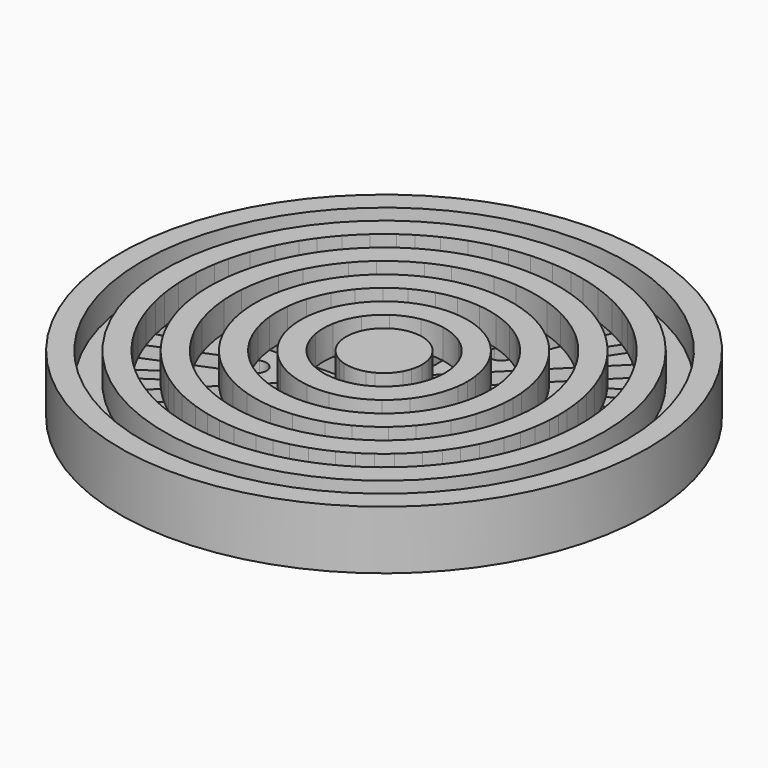
from build123d import *

# Parameters (mm, degrees)
F0_R     = 36
F1_DEPTH = 4
F2_R     = 36
F2_R_2   = 33
F2_R_3   = 30
F3_DEPTH = 4


with BuildPart() as f1:
    # F0 (on Top) → F1 (new body)
    with BuildSketch(Plane.XY):
        Circle(F0_R)
        with BuildLine():
            Line((-11.6688606306, -19.2636365098), (-14.4467117957, -23.4209845713))
            ThreePointArc((-14.4467117957, -23.4209845713), (-15.8337516411, -23.6968839506), (-16.1096510203, -22.3098441053))
            Line((-16.1096510203, -22.3098441053), (-13.3317998552, -18.1524960438))
            ThreePointArc((-13.3317998552, -18.1524960438), (-11.9447600099, -17.8765966645), (-11.6688606306, -19.2636365098))
        make_face(mode=Mode.SUBTRACT)
        with BuildLine():
            Line((-3.408746965, -22.2627591311), (-4.384198575, -27.1666855331))
            ThreePointArc((-4.384198575, -27.1666855331), (-5.5600741775, -27.9523804915), (-6.3457691358, -26.7765048891))
            Line((-6.3457691358, -26.7765048891), (-5.3703175258, -21.8725784871))
            ThreePointArc((-5.3703175258, -21.8725784871), (-4.1944419233, -21.0868835287), (-3.408746965, -22.2627591311))
        make_face(mode=Mode.SUBTRACT)
        with BuildLine():
            ThreePointArc((-6.83905821, -12.5912581897), (-4.8792137627, -11.7794640395), (-4.0674196124, -13.7393084868))
            Line((-4.0674196124, -13.7393084868), (-9.4249876655, -26.673621942))
            ThreePointArc((-9.4249876655, -26.673621942), (-11.3848321129, -27.4854160922), (-12.1966262631, -25.5255716449))
            Line((-12.1966262631, -25.5255716449), (-6.83905821, -12.5912581897))
        make_face(mode=Mode.SUBTRACT)
        with BuildLine():
            Line((-18.1524960438, -13.3317998552), (-22.3098441053, -16.1096510203))
            ThreePointArc((-22.3098441053, -16.1096510203), (-23.6968839506, -15.8337516411), (-23.4209845713, -14.4467117957))
            Line((-23.4209845713, -14.4467117957), (-19.2636365098, -11.6688606306))
            ThreePointArc((-19.2636365098, -11.6688606306), (-17.8765966645, -11.9447600099), (-18.1524960438, -13.3317998552))
        make_face(mode=Mode.SUBTRACT)
        with BuildLine():
            Line((-21.8725784871, -5.3703175258), (-26.7765048891, -6.3457691358))
            ThreePointArc((-26.7765048891, -6.3457691358), (-27.9523804915, -5.5600741775), (-27.1666855331, -4.384198575))
            Line((-27.1666855331, -4.384198575), (-22.2627591311, -3.408746965))
            ThreePointArc((-22.2627591311, -3.408746965), (-21.0868835287, -4.1944419233), (-21.8725784871, -5.3703175258))
        make_face(mode=Mode.SUBTRACT)
        with BuildLine():
            ThreePointArc((-13.7393084868, -4.0674196124), (-11.7794640395, -4.8792137627), (-12.5912581897, -6.83905821))
            Line((-12.5912581897, -6.83905821), (-25.5255716449, -12.1966262631))
            ThreePointArc((-25.5255716449, -12.1966262631), (-27.4854160922, -11.3848321129), (-26.673621942, -9.4249876655))
            Line((-26.673621942, -9.4249876655), (-13.7393084868, -4.0674196124))
        make_face(mode=Mode.SUBTRACT)
        with BuildLine():
            Line((5.3703175258, -21.8725784871), (6.3457691358, -26.7765048891))
            ThreePointArc((6.3457691358, -26.7765048891), (5.5600741775, -27.9523804915), (4.384198575, -27.1666855331))
            Line((4.384198575, -27.1666855331), (3.408746965, -22.2627591311))
            ThreePointArc((3.408746965, -22.2627591311), (4.1944419233, -21.0868835287), (5.3703175258, -21.8725784871))
        make_face(mode=Mode.SUBTRACT)
        with BuildLine():
            ThreePointArc((4.0674196124, -13.7393084868), (4.8792137627, -11.7794640395), (6.83905821, -12.5912581897))
            Line((6.83905821, -12.5912581897), (12.1966262631, -25.5255716449))
            ThreePointArc((12.1966262631, -25.5255716449), (11.3848321129, -27.4854160922), (9.4249876655, -26.673621942))
            Line((9.4249876655, -26.673621942), (4.0674196124, -13.7393084868))
        make_face(mode=Mode.SUBTRACT)
        with BuildLine():
            Line((13.3317998552, -18.1524960438), (16.1096510203, -22.3098441053))
            ThreePointArc((16.1096510203, -22.3098441053), (15.8337516411, -23.6968839506), (14.4467117957, -23.4209845713))
            Line((14.4467117957, -23.4209845713), (11.6688606306, -19.2636365098))
            ThreePointArc((11.6688606306, -19.2636365098), (11.9447600099, -17.8765966645), (13.3317998552, -18.1524960438))
        make_face(mode=Mode.SUBTRACT)
        with BuildLine():
            Line((19.2636365098, -11.6688606306), (23.4209845713, -14.4467117957))
            ThreePointArc((23.4209845713, -14.4467117957), (23.6968839506, -15.8337516411), (22.3098441053, -16.1096510203))
            Line((22.3098441053, -16.1096510203), (18.1524960438, -13.3317998552))
            ThreePointArc((18.1524960438, -13.3317998552), (17.8765966645, -11.9447600099), (19.2636365098, -11.6688606306))
        make_face(mode=Mode.SUBTRACT)
        with BuildLine():
            ThreePointArc((12.5912581897, -6.83905821), (11.7794640395, -4.8792137627), (13.7393084868, -4.0674196124))
            Line((13.7393084868, -4.0674196124), (26.673621942, -9.4249876655))
            ThreePointArc((26.673621942, -9.4249876655), (27.4854160922, -11.3848321129), (25.5255716449, -12.1966262631))
            Line((25.5255716449, -12.1966262631), (12.5912581897, -6.83905821))
        make_face(mode=Mode.SUBTRACT)
        with BuildLine():
            Line((22.2627591311, -3.408746965), (27.1666855331, -4.384198575))
            ThreePointArc((27.1666855331, -4.384198575), (27.9523804915, -5.5600741775), (26.7765048891, -6.3457691358))
            Line((26.7765048891, -6.3457691358), (21.8725784871, -5.3703175258))
            ThreePointArc((21.8725784871, -5.3703175258), (21.0868835287, -4.1944419233), (22.2627591311, -3.408746965))
        make_face(mode=Mode.SUBTRACT)
        with BuildLine():
            Line((-22.2627591311, 3.408746965), (-27.1666855331, 4.384198575))
            ThreePointArc((-27.1666855331, 4.384198575), (-27.9523804915, 5.5600741775), (-26.7765048891, 6.3457691358))
            Line((-26.7765048891, 6.3457691358), (-21.8725784871, 5.3703175258))
            ThreePointArc((-21.8725784871, 5.3703175258), (-21.0868835287, 4.1944419233), (-22.2627591311, 3.408746965))
        make_face(mode=Mode.SUBTRACT)
        with BuildLine():
            ThreePointArc((-12.5912581897, 6.83905821), (-11.7794640395, 4.8792137627), (-13.7393084868, 4.0674196124))
            Line((-13.7393084868, 4.0674196124), (-26.673621942, 9.4249876655))
            ThreePointArc((-26.673621942, 9.4249876655), (-27.4854160922, 11.3848321129), (-25.5255716449, 12.1966262631))
            Line((-25.5255716449, 12.1966262631), (-12.5912581897, 6.83905821))
        make_face(mode=Mode.SUBTRACT)
        with BuildLine():
            Line((-19.2636365098, 11.6688606306), (-23.4209845713, 14.4467117957))
            ThreePointArc((-23.4209845713, 14.4467117957), (-23.6968839506, 15.8337516411), (-22.3098441053, 16.1096510203))
            Line((-22.3098441053, 16.1096510203), (-18.1524960438, 13.3317998552))
            ThreePointArc((-18.1524960438, 13.3317998552), (-17.8765966645, 11.9447600099), (-19.2636365098, 11.6688606306))
        make_face(mode=Mode.SUBTRACT)
        with BuildLine():
            Line((-13.3317998552, 18.1524960438), (-16.1096510203, 22.3098441053))
            ThreePointArc((-16.1096510203, 22.3098441053), (-15.8337516411, 23.6968839506), (-14.4467117957, 23.4209845713))
            Line((-14.4467117957, 23.4209845713), (-11.6688606306, 19.2636365098))
            ThreePointArc((-11.6688606306, 19.2636365098), (-11.9447600099, 17.8765966645), (-13.3317998552, 18.1524960438))
        make_face(mode=Mode.SUBTRACT)
        with BuildLine():
            ThreePointArc((-4.0674196124, 13.7393084868), (-4.8792137627, 11.7794640395), (-6.83905821, 12.5912581897))
            Line((-6.83905821, 12.5912581897), (-12.1966262631, 25.5255716449))
            ThreePointArc((-12.1966262631, 25.5255716449), (-11.3848321129, 27.4854160922), (-9.4249876655, 26.673621942))
            Line((-9.4249876655, 26.673621942), (-4.0674196124, 13.7393084868))
        make_face(mode=Mode.SUBTRACT)
        with BuildLine():
            Line((-5.3703175258, 21.8725784871), (-6.3457691358, 26.7765048891))
            ThreePointArc((-6.3457691358, 26.7765048891), (-5.5600741775, 27.9523804915), (-4.384198575, 27.1666855331))
            Line((-4.384198575, 27.1666855331), (-3.408746965, 22.2627591311))
            ThreePointArc((-3.408746965, 22.2627591311), (-4.1944419233, 21.0868835287), (-5.3703175258, 21.8725784871))
        make_face(mode=Mode.SUBTRACT)
        with BuildLine():
            Line((-1.5, 3.6213203436), (-1.5, 27.5))
            ThreePointArc((-1.5, 27.5), (0, 29), (1.5, 27.5))
            Line((1.5, 27.5), (1.5, 3.6213203436))
            Line((1.5, 3.6213203436), (18.3847763109, 20.5060966544))
            ThreePointArc((18.3847763109, 20.5060966544), (20.5060966544, 20.5060966544), (20.5060966544, 18.3847763109))
            Line((20.5060966544, 18.3847763109), (3.6213203436, 1.5))
            Line((3.6213203436, 1.5), (27.5, 1.5))
            ThreePointArc((27.5, 1.5), (29, 0), (27.5, -1.5))
            Line((27.5, -1.5), (3.6213203436, -1.5))
            Line((3.6213203436, -1.5), (20.5060966544, -18.3847763109))
            ThreePointArc((20.5060966544, -18.3847763109), (20.5060966544, -20.5060966544), (18.3847763109, -20.5060966544))
            Line((18.3847763109, -20.5060966544), (1.5, -3.6213203436))
            Line((1.5, -3.6213203436), (1.5, -27.5))
            ThreePointArc((1.5, -27.5), (0, -29), (-1.5, -27.5))
            Line((-1.5, -27.5), (-1.5, -3.6213203436))
            Line((-1.5, -3.6213203436), (-18.3847763109, -20.5060966544))
            ThreePointArc((-18.3847763109, -20.5060966544), (-20.5060966544, -20.5060966544), (-20.5060966544, -18.3847763109))
            Line((-20.5060966544, -18.3847763109), (-3.6213203436, -1.5))
            Line((-3.6213203436, -1.5), (-27.5, -1.5))
            ThreePointArc((-27.5, -1.5), (-29, 0), (-27.5, 1.5))
            Line((-27.5, 1.5), (-3.6213203436, 1.5))
            Line((-3.6213203436, 1.5), (-20.5060966544, 18.3847763109))
            ThreePointArc((-20.5060966544, 18.3847763109), (-20.5060966544, 20.5060966544), (-18.3847763109, 20.5060966544))
            Line((-18.3847763109, 20.5060966544), (-1.5, 3.6213203436))
        make_face(mode=Mode.SUBTRACT)
        with BuildLine():
            ThreePointArc((13.7393084868, 4.0674196124), (11.7794640395, 4.8792137627), (12.5912581897, 6.83905821))
            Line((12.5912581897, 6.83905821), (25.5255716449, 12.1966262631))
            ThreePointArc((25.5255716449, 12.1966262631), (27.4854160922, 11.3848321129), (26.673621942, 9.4249876655))
            Line((26.673621942, 9.4249876655), (13.7393084868, 4.0674196124))
        make_face(mode=Mode.SUBTRACT)
        with BuildLine():
            Line((21.8725784871, 5.3703175258), (26.7765048891, 6.3457691358))
            ThreePointArc((26.7765048891, 6.3457691358), (27.9523804915, 5.5600741775), (27.1666855331, 4.384198575))
            Line((27.1666855331, 4.384198575), (22.2627591311, 3.408746965))
            ThreePointArc((22.2627591311, 3.408746965), (21.0868835287, 4.1944419233), (21.8725784871, 5.3703175258))
        make_face(mode=Mode.SUBTRACT)
        with BuildLine():
            Line((18.1524960438, 13.3317998552), (22.3098441053, 16.1096510203))
            ThreePointArc((22.3098441053, 16.1096510203), (23.6968839506, 15.8337516411), (23.4209845713, 14.4467117957))
            Line((23.4209845713, 14.4467117957), (19.2636365098, 11.6688606306))
            ThreePointArc((19.2636365098, 11.6688606306), (17.8765966645, 11.9447600099), (18.1524960438, 13.3317998552))
        make_face(mode=Mode.SUBTRACT)
        with BuildLine():
            Line((12.1966262631, 25.5255716449), (6.83905821, 12.5912581897))
            ThreePointArc((6.83905821, 12.5912581897), (4.8792137627, 11.7794640395), (4.0674196124, 13.7393084868))
            Line((4.0674196124, 13.7393084868), (9.4249876655, 26.673621942))
            ThreePointArc((9.4249876655, 26.673621942), (11.3848321129, 27.4854160922), (12.1966262631, 25.5255716449))
        make_face(mode=Mode.SUBTRACT)
        with BuildLine():
            Line((3.408746965, 22.2627591311), (4.384198575, 27.1666855331))
            ThreePointArc((4.384198575, 27.1666855331), (5.5600741775, 27.9523804915), (6.3457691358, 26.7765048891))
            Line((6.3457691358, 26.7765048891), (5.3703175258, 21.8725784871))
            ThreePointArc((5.3703175258, 21.8725784871), (4.1944419233, 21.0868835287), (3.408746965, 22.2627591311))
        make_face(mode=Mode.SUBTRACT)
        with BuildLine():
            Line((11.6688606306, 19.2636365098), (14.4467117957, 23.4209845713))
            ThreePointArc((14.4467117957, 23.4209845713), (15.8337516411, 23.6968839506), (16.1096510203, 22.3098441053))
            Line((16.1096510203, 22.3098441053), (13.3317998552, 18.1524960438))
            ThreePointArc((13.3317998552, 18.1524960438), (11.9447600099, 17.8765966645), (11.6688606306, 19.2636365098))
        make_face(mode=Mode.SUBTRACT)
    extrude(amount=F1_DEPTH)

    # F2 (on face) → F3 (join)
    with BuildSketch(Plane.XY.offset(4)):
        Circle(F2_R)
        Circle(F2_R_2, mode=Mode.SUBTRACT)
        Circle(F2_R_3)
        with BuildLine():
            ThreePointArc((26.5565934946, 4.2628437233), (26.7413478903, 2.8852742779), (26.8546922278, 1.5))
            Line((26.8546922278, 1.5), (27.5, 1.5))
            ThreePointArc((27.5, 1.5), (29, 0), (27.5, -1.5))
            Line((27.5, -1.5), (26.8546922278, -1.5))
            ThreePointArc((26.8546922278, -1.5), (26.7413478903, -2.8852742779), (26.5565934946, -4.2628437233))
            Line((26.5565934946, -4.2628437233), (27.1666855331, -4.384198575))
            ThreePointArc((27.1666855331, -4.384198575), (27.9523804915, -5.5600741775), (26.7765048891, -6.3457691358))
            Line((26.7765048891, -6.3457691358), (26.1664128506, -6.2244142842))
            ThreePointArc((26.1664128506, -6.2244142842), (25.8099306516, -7.5678249457), (25.3845256497, -8.8910264981))
            Line((25.3845256497, -8.8910264981), (26.673621942, -9.4249876655))
            ThreePointArc((26.673621942, -9.4249876655), (27.4854160922, -11.3848321129), (25.5255716449, -12.1966262631))
            Line((25.5255716449, -12.1966262631), (24.2364753526, -11.6626650956))
            ThreePointArc((24.2364753526, -11.6626650956), (23.6016373236, -12.8991166478), (22.9037735152, -14.1011224168))
            Line((22.9037735152, -14.1011224168), (23.4209845713, -14.4467117957))
            ThreePointArc((23.4209845713, -14.4467117957), (23.6968839506, -15.8337516411), (22.3098441053, -16.1096510203))
            Line((22.3098441053, -16.1096510203), (21.7926330492, -15.7640616414))
            ThreePointArc((21.7926330492, -15.7640616414), (20.9491854388, -16.8687914238), (20.0497951527, -17.9284748092))
            Line((20.0497951527, -17.9284748092), (20.5060966544, -18.3847763109))
            ThreePointArc((20.5060966544, -18.3847763109), (20.5060966544, -20.5060966544), (18.3847763109, -20.5060966544))
            Line((18.3847763109, -20.5060966544), (17.9284748092, -20.0497951527))
            ThreePointArc((17.9284748092, -20.0497951527), (16.8687914238, -20.9491854388), (15.7640616414, -21.7926330492))
            Line((15.7640616414, -21.7926330492), (16.1096510203, -22.3098441053))
            ThreePointArc((16.1096510203, -22.3098441053), (15.8337516411, -23.6968839506), (14.4467117957, -23.4209845713))
            Line((14.4467117957, -23.4209845713), (14.1011224167, -22.9037735152))
            ThreePointArc((14.1011224168, -22.9037735152), (12.8991166478, -23.6016373236), (11.6626650956, -24.2364753526))
            Line((11.6626650956, -24.2364753526), (12.1966262631, -25.5255716449))
            ThreePointArc((12.1966262631, -25.5255716449), (11.3848321129, -27.4854160922), (9.4249876655, -26.673621942))
            Line((9.4249876655, -26.673621942), (8.8910264981, -25.3845256497))
            ThreePointArc((8.8910264981, -25.3845256497), (7.5678249457, -25.8099306516), (6.2244142842, -26.1664128506))
            Line((6.2244142842, -26.1664128506), (6.3457691358, -26.7765048891))
            ThreePointArc((6.3457691358, -26.7765048891), (5.5600741775, -27.9523804915), (4.384198575, -27.1666855331))
            Line((4.384198575, -27.1666855331), (4.2628437233, -26.5565934946))
            ThreePointArc((4.2628437233, -26.5565934946), (2.8852742779, -26.7413478903), (1.5, -26.8546922278))
            Line((1.5, -26.8546922278), (1.5, -27.5))
            ThreePointArc((1.5, -27.5), (0, -29), (-1.5, -27.5))
            Line((-1.5, -27.5), (-1.5, -26.8546922278))
            ThreePointArc((-1.5, -26.8546922278), (-2.8852742779, -26.7413478903), (-4.2628437233, -26.5565934946))
            Line((-4.2628437233, -26.5565934946), (-4.384198575, -27.1666855331))
            ThreePointArc((-4.384198575, -27.1666855331), (-5.5600741775, -27.9523804915), (-6.3457691358, -26.7765048891))
            Line((-6.3457691358, -26.7765048891), (-6.2244142842, -26.1664128506))
            ThreePointArc((-6.2244142842, -26.1664128506), (-7.5678249457, -25.8099306516), (-8.8910264981, -25.3845256497))
            Line((-8.8910264981, -25.3845256497), (-9.4249876655, -26.673621942))
            ThreePointArc((-9.4249876655, -26.673621942), (-11.3848321129, -27.4854160922), (-12.1966262631, -25.5255716449))
            Line((-12.1966262631, -25.5255716449), (-11.6626650956, -24.2364753526))
            ThreePointArc((-11.6626650956, -24.2364753526), (-12.8991166478, -23.6016373236), (-14.1011224168, -22.9037735152))
            Line((-14.1011224168, -22.9037735152), (-14.4467117957, -23.4209845713))
            ThreePointArc((-14.4467117957, -23.4209845713), (-15.8337516411, -23.6968839506), (-16.1096510203, -22.3098441053))
            Line((-16.1096510203, -22.3098441053), (-15.7640616414, -21.7926330492))
            ThreePointArc((-15.7640616414, -21.7926330492), (-16.8687914238, -20.9491854388), (-17.9284748092, -20.0497951527))
            Line((-17.9284748092, -20.0497951527), (-18.3847763109, -20.5060966544))
            ThreePointArc((-18.3847763109, -20.5060966544), (-20.5060966544, -20.5060966544), (-20.5060966544, -18.3847763109))
            Line((-20.5060966544, -18.3847763109), (-20.0497951527, -17.9284748092))
            ThreePointArc((-20.0497951527, -17.9284748092), (-20.9491854388, -16.8687914238), (-21.7926330492, -15.7640616414))
            Line((-21.7926330492, -15.7640616414), (-22.3098441053, -16.1096510203))
            ThreePointArc((-22.3098441053, -16.1096510203), (-23.6968839506, -15.8337516411), (-23.4209845713, -14.4467117957))
            Line((-23.4209845713, -14.4467117957), (-22.9037735152, -14.1011224167))
            ThreePointArc((-22.9037735152, -14.1011224168), (-23.6016373236, -12.8991166478), (-24.2364753526, -11.6626650956))
            Line((-24.2364753526, -11.6626650956), (-25.5255716449, -12.1966262631))
            ThreePointArc((-25.5255716449, -12.1966262631), (-27.4854160922, -11.3848321129), (-26.673621942, -9.4249876655))
            Line((-26.673621942, -9.4249876655), (-25.3845256497, -8.8910264981))
            ThreePointArc((-25.3845256497, -8.8910264981), (-25.8099306516, -7.5678249457), (-26.1664128506, -6.2244142842))
            Line((-26.1664128506, -6.2244142842), (-26.7765048891, -6.3457691358))
            ThreePointArc((-26.7765048891, -6.3457691358), (-27.9523804915, -5.5600741775), (-27.1666855331, -4.384198575))
            Line((-27.1666855331, -4.384198575), (-26.5565934946, -4.2628437233))
            ThreePointArc((-26.5565934946, -4.2628437233), (-26.7413478903, -2.8852742779), (-26.8546922278, -1.5))
            Line((-26.8546922278, -1.5), (-27.5, -1.5))
            ThreePointArc((-27.5, -1.5), (-29, 0), (-27.5, 1.5))
            Line((-27.5, 1.5), (-26.8546922278, 1.5))
            ThreePointArc((-26.8546922278, 1.5), (-26.7413478903, 2.8852742779), (-26.5565934946, 4.2628437233))
            Line((-26.5565934946, 4.2628437233), (-27.1666855331, 4.384198575))
            ThreePointArc((-27.1666855331, 4.384198575), (-27.9523804915, 5.5600741775), (-26.7765048891, 6.3457691358))
            Line((-26.7765048891, 6.3457691358), (-26.1664128506, 6.2244142842))
            ThreePointArc((-26.1664128506, 6.2244142842), (-25.8099306516, 7.5678249457), (-25.3845256497, 8.8910264981))
            Line((-25.3845256497, 8.8910264981), (-26.673621942, 9.4249876655))
            ThreePointArc((-26.673621942, 9.4249876655), (-27.4854160922, 11.3848321129), (-25.5255716449, 12.1966262631))
            Line((-25.5255716449, 12.1966262631), (-24.2364753526, 11.6626650956))
            ThreePointArc((-24.2364753526, 11.6626650956), (-23.6016373236, 12.8991166478), (-22.9037735152, 14.1011224168))
            Line((-22.9037735152, 14.1011224168), (-23.4209845713, 14.4467117957))
            ThreePointArc((-23.4209845713, 14.4467117957), (-23.6968839506, 15.8337516411), (-22.3098441053, 16.1096510203))
            Line((-22.3098441053, 16.1096510203), (-21.7926330492, 15.7640616414))
            ThreePointArc((-21.7926330492, 15.7640616414), (-20.9491854388, 16.8687914238), (-20.0497951527, 17.9284748092))
            Line((-20.0497951527, 17.9284748092), (-20.5060966544, 18.3847763109))
            ThreePointArc((-20.5060966544, 18.3847763109), (-20.5060966544, 20.5060966544), (-18.3847763109, 20.5060966544))
            Line((-18.3847763109, 20.5060966544), (-17.9284748092, 20.0497951527))
            ThreePointArc((-17.9284748092, 20.0497951527), (-16.8687914238, 20.9491854388), (-15.7640616414, 21.7926330492))
            Line((-15.7640616414, 21.7926330492), (-16.1096510203, 22.3098441053))
            ThreePointArc((-16.1096510203, 22.3098441053), (-15.8337516411, 23.6968839506), (-14.4467117957, 23.4209845713))
            Line((-14.4467117957, 23.4209845713), (-14.1011224167, 22.9037735152))
            ThreePointArc((-14.1011224168, 22.9037735152), (-12.8991166478, 23.6016373236), (-11.6626650956, 24.2364753526))
            Line((-11.6626650956, 24.2364753526), (-12.1966262631, 25.5255716449))
            ThreePointArc((-12.1966262631, 25.5255716449), (-11.3848321129, 27.4854160922), (-9.4249876655, 26.673621942))
            Line((-9.4249876655, 26.673621942), (-8.8910264981, 25.3845256497))
            ThreePointArc((-8.8910264981, 25.3845256497), (-7.5678249457, 25.8099306516), (-6.2244142842, 26.1664128506))
            Line((-6.2244142842, 26.1664128506), (-6.3457691358, 26.7765048891))
            ThreePointArc((-6.3457691358, 26.7765048891), (-5.5600741775, 27.9523804915), (-4.384198575, 27.1666855331))
            Line((-4.384198575, 27.1666855331), (-4.2628437233, 26.5565934946))
            ThreePointArc((-4.2628437233, 26.5565934946), (-2.8852742779, 26.7413478903), (-1.5, 26.8546922278))
            Line((-1.5, 26.8546922278), (-1.5, 27.5))
            ThreePointArc((-1.5, 27.5), (0, 29), (1.5, 27.5))
            Line((1.5, 27.5), (1.5, 26.8546922278))
            ThreePointArc((1.5, 26.8546922278), (2.8852742779, 26.7413478903), (4.2628437233, 26.5565934946))
            Line((4.2628437233, 26.5565934946), (4.384198575, 27.1666855331))
            ThreePointArc((4.384198575, 27.1666855331), (5.5600741775, 27.9523804915), (6.3457691358, 26.7765048891))
            Line((6.3457691358, 26.7765048891), (6.2244142842, 26.1664128506))
            ThreePointArc((6.2244142842, 26.1664128506), (7.5678249457, 25.8099306516), (8.8910264981, 25.3845256497))
            Line((8.8910264981, 25.3845256497), (9.4249876655, 26.673621942))
            ThreePointArc((9.4249876655, 26.673621942), (11.3848321129, 27.4854160922), (12.1966262631, 25.5255716449))
            Line((12.1966262631, 25.5255716449), (11.6626650956, 24.2364753526))
            ThreePointArc((11.6626650956, 24.2364753526), (12.8991166478, 23.6016373236), (14.1011224168, 22.9037735152))
            Line((14.1011224168, 22.9037735152), (14.4467117957, 23.4209845713))
            ThreePointArc((14.4467117957, 23.4209845713), (15.8337516411, 23.6968839506), (16.1096510203, 22.3098441053))
            Line((16.1096510203, 22.3098441053), (15.7640616414, 21.7926330492))
            ThreePointArc((15.7640616414, 21.7926330492), (16.8687914238, 20.9491854388), (17.9284748092, 20.0497951527))
            Line((17.9284748092, 20.0497951527), (18.3847763109, 20.5060966544))
            ThreePointArc((18.3847763109, 20.5060966544), (20.5060966544, 20.5060966544), (20.5060966544, 18.3847763109))
            Line((20.5060966544, 18.3847763109), (20.0497951527, 17.9284748092))
            ThreePointArc((20.0497951527, 17.9284748092), (20.9491854388, 16.8687914238), (21.7926330492, 15.7640616414))
            Line((21.7926330492, 15.7640616414), (22.3098441053, 16.1096510203))
            ThreePointArc((22.3098441053, 16.1096510203), (23.6968839506, 15.8337516411), (23.4209845713, 14.4467117957))
            Line((23.4209845713, 14.4467117957), (22.9037735152, 14.1011224167))
            ThreePointArc((22.9037735152, 14.1011224168), (23.6016373236, 12.8991166478), (24.2364753526, 11.6626650956))
            Line((24.2364753526, 11.6626650956), (25.5255716449, 12.1966262631))
            ThreePointArc((25.5255716449, 12.1966262631), (27.4854160922, 11.3848321129), (26.673621942, 9.4249876655))
            Line((26.673621942, 9.4249876655), (25.3845256497, 8.8910264981))
            ThreePointArc((25.3845256497, 8.8910264981), (25.8099306516, 7.5678249457), (26.1664128506, 6.2244142842))
            Line((26.1664128506, 6.2244142842), (26.7765048891, 6.3457691358))
            ThreePointArc((26.7765048891, 6.3457691358), (27.9523804915, 5.5600741775), (27.1666855331, 4.384198575))
            Line((27.1666855331, 4.384198575), (26.5565934946, 4.2628437233))
        make_face(mode=Mode.SUBTRACT)
        with BuildLine():
            ThreePointArc((5.1724137931, 0), (5.1165430512, 0.7581897203), (4.950137821, 1.5))
            Line((4.950137821, 1.5), (3.6213203436, 1.5))
            Line((3.6213203436, 1.5), (4.5609361928, 2.4396158493))
            ThreePointArc((4.5609361928, 2.4396158493), (3.6574488682, 3.6574488682), (2.4396158493, 4.5609361928))
            Line((2.4396158493, 4.5609361928), (1.5, 3.6213203436))
            Line((1.5, 3.6213203436), (1.5, 4.950137821))
            ThreePointArc((1.5, 4.950137821), (0, 5.1724137931), (-1.5, 4.950137821))
            Line((-1.5, 4.950137821), (-1.5, 3.6213203436))
            Line((-1.5, 3.6213203436), (-2.4396158493, 4.5609361928))
            ThreePointArc((-2.4396158493, 4.5609361928), (-3.6574488682, 3.6574488682), (-4.5609361928, 2.4396158493))
            Line((-4.5609361928, 2.4396158493), (-3.6213203436, 1.5))
            Line((-3.6213203436, 1.5), (-4.950137821, 1.5))
            ThreePointArc((-4.950137821, 1.5), (-5.1724137931, 0), (-4.950137821, -1.5))
            Line((-4.950137821, -1.5), (-3.6213203436, -1.5))
            Line((-3.6213203436, -1.5), (-4.5609361928, -2.4396158493))
            ThreePointArc((-4.5609361928, -2.4396158493), (-3.6574488682, -3.6574488682), (-2.4396158493, -4.5609361928))
            Line((-2.4396158493, -4.5609361928), (-1.5, -3.6213203436))
            Line((-1.5, -3.6213203436), (-1.5, -4.950137821))
            ThreePointArc((-1.5, -4.950137821), (0, -5.1724137931), (1.5, -4.950137821))
            Line((1.5, -4.950137821), (1.5, -3.6213203436))
            Line((1.5, -3.6213203436), (2.4396158493, -4.5609361928))
            ThreePointArc((2.4396158493, -4.5609361928), (3.6574488682, -3.6574488682), (4.5609361928, -2.4396158493))
            Line((4.5609361928, -2.4396158493), (3.6213203436, -1.5))
            Line((3.6213203436, -1.5), (4.950137821, -1.5))
            ThreePointArc((4.950137821, -1.5), (5.1165430512, -0.7581897203), (5.1724137931, 0))
        make_face()
        with BuildLine():
            Line((8.1387894053, 1.5), (11.2800134718, 1.5))
            ThreePointArc((11.2800134718, 1.5), (10.5131119217, 4.3546735407), (9.0368341896, 6.915513846))
            Line((9.0368341896, 6.915513846), (6.8156533509, 4.6943330074))
            ThreePointArc((6.8156533509, 4.6943330074), (7.6458995794, 3.1670353023), (8.1387894053, 1.5))
        make_face()
        with BuildLine():
            ThreePointArc((9.0368341896, -6.915513846), (10.5131119217, -4.3546735407), (11.2800134718, -1.5))
            Line((11.2800134718, -1.5), (8.1387894053, -1.5))
            ThreePointArc((8.1387894053, -1.5), (7.6458995794, -3.1670353023), (6.8156533509, -4.6943330074))
            Line((6.8156533509, -4.6943330074), (9.0368341896, -6.915513846))
        make_face()
        with BuildLine():
            ThreePointArc((1.5, -11.2800134718), (4.3546735407, -10.5131119217), (6.915513846, -9.0368341896))
            Line((6.915513846, -9.0368341896), (4.6943330074, -6.8156533509))
            ThreePointArc((4.6943330074, -6.8156533509), (3.1670353023, -7.6458995794), (1.5, -8.1387894053))
            Line((1.5, -8.1387894053), (1.5, -11.2800134718))
        make_face()
        with BuildLine():
            ThreePointArc((-6.915513846, -9.0368341896), (-4.3546735407, -10.5131119217), (-1.5, -11.2800134718))
            Line((-1.5, -11.2800134718), (-1.5, -8.1387894053))
            ThreePointArc((-1.5, -8.1387894053), (-3.1670353023, -7.6458995794), (-4.6943330074, -6.8156533509))
            Line((-4.6943330074, -6.8156533509), (-6.915513846, -9.0368341896))
        make_face()
        with BuildLine():
            ThreePointArc((-11.2800134718, -1.5), (-10.5131119217, -4.3546735407), (-9.0368341896, -6.915513846))
            Line((-9.0368341896, -6.915513846), (-6.8156533509, -4.6943330074))
            ThreePointArc((-6.8156533509, -4.6943330074), (-7.6458995794, -3.1670353023), (-8.1387894053, -1.5))
            Line((-8.1387894053, -1.5), (-11.2800134718, -1.5))
        make_face()
        with BuildLine():
            Line((-6.8156533509, 4.6943330074), (-9.0368341896, 6.915513846))
            ThreePointArc((-9.0368341896, 6.915513846), (-10.5131119217, 4.3546735407), (-11.2800134718, 1.5))
            Line((-11.2800134718, 1.5), (-8.1387894053, 1.5))
            ThreePointArc((-8.1387894053, 1.5), (-7.6458995794, 3.1670353023), (-6.8156533509, 4.6943330074))
        make_face()
        with BuildLine():
            Line((-1.5, 8.1387894053), (-1.5, 11.2800134718))
            ThreePointArc((-1.5, 11.2800134718), (-4.3546735407, 10.5131119217), (-6.915513846, 9.0368341896))
            Line((-6.915513846, 9.0368341896), (-4.6943330074, 6.8156533509))
            ThreePointArc((-4.6943330074, 6.8156533509), (-3.1670353023, 7.6458995794), (-1.5, 8.1387894053))
        make_face()
        with BuildLine():
            Line((4.6943330074, 6.8156533509), (6.915513846, 9.0368341896))
            ThreePointArc((6.915513846, 9.0368341896), (4.3546735407, 10.5131119217), (1.5, 11.2800134718))
            Line((1.5, 11.2800134718), (1.5, 8.1387894053))
            ThreePointArc((1.5, 8.1387894053), (3.1670353023, 7.6458995794), (4.6943330074, 6.8156533509))
        make_face()
        with BuildLine():
            ThreePointArc((9.2825717273, 18.4904216631), (11.4945565452, 17.2028195649), (13.5306357123, 15.6519560559))
            Line((13.5306357123, 15.6519560559), (15.730137482, 17.8514578256))
            ThreePointArc((15.730137482, 17.8514578256), (14.8998296014, 18.5501172382), (14.0385294523, 19.2101916314))
            Line((14.0385294523, 19.2101916314), (13.3317998552, 18.1524960438))
            ThreePointArc((13.3317998552, 18.1524960438), (11.9447600099, 17.8765966645), (11.6688606306, 19.2636365098))
            Line((11.6688606306, 19.2636365098), (12.3755902277, 20.3213320975))
            ThreePointArc((12.3755902277, 20.3213320975), (11.4361557085, 20.8644701421), (10.4729335073, 21.3642092166))
            Line((10.4729335073, 21.3642092166), (9.2825717273, 18.4904216631))
        make_face()
        with BuildLine():
            ThreePointArc((15.6519560559, 13.5306357123), (17.2028195649, 11.4945565452), (18.4904216631, 9.2825717273))
            Line((18.4904216631, 9.2825717273), (21.3642092166, 10.4729335073))
            ThreePointArc((21.3642092166, 10.4729335073), (20.8644701421, 11.4361557085), (20.3213320975, 12.3755902277))
            Line((20.3213320975, 12.3755902277), (19.2636365098, 11.6688606306))
            ThreePointArc((19.2636365098, 11.6688606306), (17.8765966645, 11.9447600099), (18.1524960438, 13.3317998552))
            Line((18.1524960438, 13.3317998552), (19.2101916314, 14.0385294523))
            ThreePointArc((19.2101916314, 14.0385294523), (18.5501172382, 14.8998296014), (17.8514578256, 15.730137482))
            Line((17.8514578256, 15.730137482), (15.6519560559, 13.5306357123))
        make_face()
        with BuildLine():
            Line((20.6352085319, 1.5), (23.745773765, 1.5))
            ThreePointArc((23.745773765, 1.5), (23.6526842406, 2.5811431412), (23.5103961441, 3.6569173968))
            Line((23.5103961441, 3.6569173969), (22.2627591311, 3.408746965))
            ThreePointArc((22.2627591311, 3.408746965), (21.0868835287, 4.1944419233), (21.8725784871, 5.3703175258))
            Line((21.8725784871, 5.3703175258), (23.1202155001, 5.6184879577))
            ThreePointArc((23.1202155001, 5.6184879577), (22.8399915755, 6.6668250712), (22.5122595137, 7.7012949098))
            Line((22.5122595137, 7.7012949098), (19.6384719602, 6.5109331298))
            ThreePointArc((19.6384719602, 6.5109331298), (20.2921092497, 4.03635149), (20.6352085319, 1.5))
        make_face()
        with BuildLine():
            ThreePointArc((23.5103961441, -3.6569173968), (23.6526842406, -2.5811431412), (23.745773765, -1.5))
            Line((23.745773765, -1.5), (20.6352085319, -1.5))
            ThreePointArc((20.6352085319, -1.5), (20.2921092497, -4.03635149), (19.6384719602, -6.5109331298))
            Line((19.6384719602, -6.5109331298), (22.5122595137, -7.7012949098))
            ThreePointArc((22.5122595137, -7.7012949098), (22.8399915755, -6.6668250712), (23.1202155001, -5.6184879577))
            Line((23.1202155001, -5.6184879577), (21.8725784871, -5.3703175258))
            ThreePointArc((21.8725784871, -5.3703175258), (21.0868835287, -4.1944419233), (22.2627591311, -3.408746965))
            Line((22.2627591311, -3.408746965), (23.5103961441, -3.6569173969))
        make_face()
        with BuildLine():
            Line((21.3642092166, -10.4729335073), (18.4904216631, -9.2825717273))
            ThreePointArc((18.4904216631, -9.2825717273), (17.2028195649, -11.4945565452), (15.6519560559, -13.5306357123))
            Line((15.6519560559, -13.5306357123), (17.8514578256, -15.730137482))
            ThreePointArc((17.8514578256, -15.730137482), (18.5501172382, -14.8998296014), (19.2101916314, -14.0385294523))
            Line((19.2101916314, -14.0385294523), (18.1524960438, -13.3317998552))
            ThreePointArc((18.1524960438, -13.3317998552), (17.8765966645, -11.9447600099), (19.2636365098, -11.6688606306))
            Line((19.2636365098, -11.6688606306), (20.3213320975, -12.3755902277))
            ThreePointArc((20.3213320975, -12.3755902277), (20.8644701421, -11.4361557085), (21.3642092166, -10.4729335073))
        make_face()
        with BuildLine():
            Line((15.730137482, -17.8514578256), (13.5306357123, -15.6519560559))
            ThreePointArc((13.5306357123, -15.6519560559), (11.4945565452, -17.2028195649), (9.2825717273, -18.4904216631))
            Line((9.2825717273, -18.4904216631), (10.4729335073, -21.3642092166))
            ThreePointArc((10.4729335073, -21.3642092166), (11.4361557085, -20.8644701421), (12.3755902277, -20.3213320975))
            Line((12.3755902277, -20.3213320975), (11.6688606306, -19.2636365098))
            ThreePointArc((11.6688606306, -19.2636365098), (11.9447600099, -17.8765966645), (13.3317998552, -18.1524960438))
            Line((13.3317998552, -18.1524960438), (14.0385294523, -19.2101916314))
            ThreePointArc((14.0385294523, -19.2101916314), (14.8998296014, -18.5501172382), (15.730137482, -17.8514578256))
        make_face()
        with BuildLine():
            Line((7.7012949098, -22.5122595137), (6.5109331298, -19.6384719602))
            ThreePointArc((6.5109331298, -19.6384719602), (4.03635149, -20.2921092497), (1.5, -20.6352085319))
            Line((1.5, -20.6352085319), (1.5, -23.745773765))
            ThreePointArc((1.5, -23.745773765), (2.5811431412, -23.6526842406), (3.6569173968, -23.5103961441))
            Line((3.6569173969, -23.5103961441), (3.408746965, -22.2627591311))
            ThreePointArc((3.408746965, -22.2627591311), (4.1944419233, -21.0868835287), (5.3703175258, -21.8725784871))
            Line((5.3703175258, -21.8725784871), (5.6184879577, -23.1202155001))
            ThreePointArc((5.6184879577, -23.1202155001), (6.6668250712, -22.8399915755), (7.7012949098, -22.5122595137))
        make_face()
        with BuildLine():
            Line((-1.5, -23.745773765), (-1.5, -20.6352085319))
            ThreePointArc((-1.5, -20.6352085319), (-4.03635149, -20.2921092497), (-6.5109331298, -19.6384719602))
            Line((-6.5109331298, -19.6384719602), (-7.7012949098, -22.5122595137))
            ThreePointArc((-7.7012949098, -22.5122595137), (-6.6668250712, -22.8399915755), (-5.6184879577, -23.1202155001))
            Line((-5.6184879577, -23.1202155001), (-5.3703175258, -21.8725784871))
            ThreePointArc((-5.3703175258, -21.8725784871), (-4.1944419233, -21.0868835287), (-3.408746965, -22.2627591311))
            Line((-3.408746965, -22.2627591311), (-3.6569173969, -23.5103961441))
            ThreePointArc((-3.6569173968, -23.5103961441), (-2.5811431412, -23.6526842406), (-1.5, -23.745773765))
        make_face()
        with BuildLine():
            Line((-10.4729335073, -21.3642092166), (-9.2825717273, -18.4904216631))
            ThreePointArc((-9.2825717273, -18.4904216631), (-11.4945565452, -17.2028195649), (-13.5306357123, -15.6519560559))
            Line((-13.5306357123, -15.6519560559), (-15.730137482, -17.8514578256))
            ThreePointArc((-15.730137482, -17.8514578256), (-14.8998296014, -18.5501172382), (-14.0385294523, -19.2101916314))
            Line((-14.0385294523, -19.2101916314), (-13.3317998552, -18.1524960438))
            ThreePointArc((-13.3317998552, -18.1524960438), (-11.9447600099, -17.8765966645), (-11.6688606306, -19.2636365098))
            Line((-11.6688606306, -19.2636365098), (-12.3755902277, -20.3213320975))
            ThreePointArc((-12.3755902277, -20.3213320975), (-11.4361557085, -20.8644701421), (-10.4729335073, -21.3642092166))
        make_face()
        with BuildLine():
            Line((-17.8514578256, -15.730137482), (-15.6519560559, -13.5306357123))
            ThreePointArc((-15.6519560559, -13.5306357123), (-17.2028195649, -11.4945565452), (-18.4904216631, -9.2825717273))
            Line((-18.4904216631, -9.2825717273), (-21.3642092166, -10.4729335073))
            ThreePointArc((-21.3642092166, -10.4729335073), (-20.8644701421, -11.4361557085), (-20.3213320975, -12.3755902277))
            Line((-20.3213320975, -12.3755902277), (-19.2636365098, -11.6688606306))
            ThreePointArc((-19.2636365098, -11.6688606306), (-17.8765966645, -11.9447600099), (-18.1524960438, -13.3317998552))
            Line((-18.1524960438, -13.3317998552), (-19.2101916314, -14.0385294523))
            ThreePointArc((-19.2101916314, -14.0385294523), (-18.5501172382, -14.8998296014), (-17.8514578256, -15.730137482))
        make_face()
        with BuildLine():
            ThreePointArc((-19.6384719602, -6.5109331298), (-20.2921092497, -4.03635149), (-20.6352085319, -1.5))
            Line((-20.6352085319, -1.5), (-23.745773765, -1.5))
            ThreePointArc((-23.745773765, -1.5), (-23.6526842406, -2.5811431412), (-23.5103961441, -3.6569173968))
            Line((-23.5103961441, -3.6569173969), (-22.2627591311, -3.408746965))
            ThreePointArc((-22.2627591311, -3.408746965), (-21.0868835287, -4.1944419233), (-21.8725784871, -5.3703175258))
            Line((-21.8725784871, -5.3703175258), (-23.1202155001, -5.6184879577))
            ThreePointArc((-23.1202155001, -5.6184879577), (-22.8399915755, -6.6668250712), (-22.5122595137, -7.7012949098))
            Line((-22.5122595137, -7.7012949098), (-19.6384719602, -6.5109331298))
        make_face()
        with BuildLine():
            Line((-23.745773765, 1.5), (-20.6352085319, 1.5))
            ThreePointArc((-20.6352085319, 1.5), (-20.2921092497, 4.03635149), (-19.6384719602, 6.5109331298))
            Line((-19.6384719602, 6.5109331298), (-22.5122595137, 7.7012949098))
            ThreePointArc((-22.5122595137, 7.7012949098), (-22.8399915755, 6.6668250712), (-23.1202155001, 5.6184879577))
            Line((-23.1202155001, 5.6184879577), (-21.8725784871, 5.3703175258))
            ThreePointArc((-21.8725784871, 5.3703175258), (-21.0868835287, 4.1944419233), (-22.2627591311, 3.408746965))
            Line((-22.2627591311, 3.408746965), (-23.5103961441, 3.6569173969))
            ThreePointArc((-23.5103961441, 3.6569173968), (-23.6526842406, 2.5811431412), (-23.745773765, 1.5))
        make_face()
        with BuildLine():
            ThreePointArc((-18.4904216631, 9.2825717273), (-17.2028195649, 11.4945565452), (-15.6519560559, 13.5306357123))
            Line((-15.6519560559, 13.5306357123), (-17.8514578256, 15.730137482))
            ThreePointArc((-17.8514578256, 15.730137482), (-18.5501172382, 14.8998296014), (-19.2101916314, 14.0385294523))
            Line((-19.2101916314, 14.0385294523), (-18.1524960438, 13.3317998552))
            ThreePointArc((-18.1524960438, 13.3317998552), (-17.8765966645, 11.9447600099), (-19.2636365098, 11.6688606306))
            Line((-19.2636365098, 11.6688606306), (-20.3213320975, 12.3755902277))
            ThreePointArc((-20.3213320975, 12.3755902277), (-20.8644701421, 11.4361557085), (-21.3642092166, 10.4729335073))
            Line((-21.3642092166, 10.4729335073), (-18.4904216631, 9.2825717273))
        make_face()
        with BuildLine():
            ThreePointArc((-13.5306357123, 15.6519560559), (-11.4945565452, 17.2028195649), (-9.2825717273, 18.4904216631))
            Line((-9.2825717273, 18.4904216631), (-10.4729335073, 21.3642092166))
            ThreePointArc((-10.4729335073, 21.3642092166), (-11.4361557085, 20.8644701421), (-12.3755902277, 20.3213320975))
            Line((-12.3755902277, 20.3213320975), (-11.6688606306, 19.2636365098))
            ThreePointArc((-11.6688606306, 19.2636365098), (-11.9447600099, 17.8765966645), (-13.3317998552, 18.1524960438))
            Line((-13.3317998552, 18.1524960438), (-14.0385294523, 19.2101916314))
            ThreePointArc((-14.0385294523, 19.2101916314), (-14.8998296014, 18.5501172382), (-15.730137482, 17.8514578256))
            Line((-15.730137482, 17.8514578256), (-13.5306357123, 15.6519560559))
        make_face()
        with BuildLine():
            ThreePointArc((-6.5109331298, 19.6384719602), (-4.03635149, 20.2921092497), (-1.5, 20.6352085319))
            Line((-1.5, 20.6352085319), (-1.5, 23.745773765))
            ThreePointArc((-1.5, 23.745773765), (-2.5811431412, 23.6526842406), (-3.6569173968, 23.5103961441))
            Line((-3.6569173969, 23.5103961441), (-3.408746965, 22.2627591311))
            ThreePointArc((-3.408746965, 22.2627591311), (-4.1944419233, 21.0868835287), (-5.3703175258, 21.8725784871))
            Line((-5.3703175258, 21.8725784871), (-5.6184879577, 23.1202155001))
            ThreePointArc((-5.6184879577, 23.1202155001), (-6.6668250712, 22.8399915755), (-7.7012949098, 22.5122595137))
            Line((-7.7012949098, 22.5122595137), (-6.5109331298, 19.6384719602))
        make_face()
        with BuildLine():
            ThreePointArc((1.5, 20.6352085319), (4.03635149, 20.2921092497), (6.5109331298, 19.6384719602))
            Line((6.5109331298, 19.6384719602), (7.7012949098, 22.5122595137))
            ThreePointArc((7.7012949098, 22.5122595137), (6.6668250712, 22.8399915755), (5.6184879577, 23.1202155001))
            Line((5.6184879577, 23.1202155001), (5.3703175258, 21.8725784871))
            ThreePointArc((5.3703175258, 21.8725784871), (4.1944419233, 21.0868835287), (3.408746965, 22.2627591311))
            Line((3.408746965, 22.2627591311), (3.6569173969, 23.5103961441))
            ThreePointArc((3.6569173968, 23.5103961441), (2.5811431412, 23.6526842406), (1.5, 23.745773765))
            Line((1.5, 23.745773765), (1.5, 20.6352085319))
        make_face()
        with BuildLine():
            Line((14.4048706091, 1.5), (17.5221195353, 1.5))
            ThreePointArc((17.5221195353, 1.5), (17.2482928623, 3.4308987665), (16.7623527534, 5.3196055473))
            Line((16.7623527534, 5.3196055473), (13.8823902728, 4.1266860287))
            ThreePointArc((13.8823902728, 4.1266860287), (14.2044764748, 2.825446043), (14.4048706091, 1.5))
        make_face()
        with BuildLine():
            ThreePointArc((16.7623527534, -5.3196055473), (17.2482928623, -3.4308987665), (17.5221195353, -1.5))
            Line((17.5221195353, -1.5), (14.4048706091, -1.5))
            ThreePointArc((14.4048706091, -1.5), (14.2044764748, -2.825446043), (13.8823902728, -4.1266860287))
            Line((13.8823902728, -4.1266860287), (16.7623527534, -5.3196055473))
        make_face()
        with BuildLine():
            ThreePointArc((13.4506697159, -11.3293493724), (14.6223966301, -9.7703730634), (15.6143024563, -8.0912441448))
            Line((15.6143024563, -8.0912441448), (12.7343399757, -6.8983246262))
            ThreePointArc((12.7343399757, -6.8983246262), (12.0419736954, -8.0461895817), (11.2464418616, -9.125121518))
            Line((11.2464418616, -9.125121518), (13.4506697159, -11.3293493724))
        make_face()
        with BuildLine():
            ThreePointArc((8.0912441448, -15.6143024563), (9.7703730634, -14.6223966301), (11.3293493724, -13.4506697159))
            Line((11.3293493724, -13.4506697159), (9.125121518, -11.2464418616))
            ThreePointArc((9.125121518, -11.2464418616), (8.0461895817, -12.0419736954), (6.8983246262, -12.7343399757))
            Line((6.8983246262, -12.7343399757), (8.0912441448, -15.6143024563))
        make_face()
        with BuildLine():
            ThreePointArc((1.5, -17.5221195353), (3.4308987665, -17.2482928623), (5.3196055473, -16.7623527534))
            Line((5.3196055473, -16.7623527534), (4.1266860287, -13.8823902728))
            ThreePointArc((4.1266860287, -13.8823902728), (2.825446043, -14.2044764748), (1.5, -14.4048706091))
            Line((1.5, -14.4048706091), (1.5, -17.5221195353))
        make_face()
        with BuildLine():
            Line((-1.5, -17.5221195353), (-1.5, -14.4048706091))
            ThreePointArc((-1.5, -14.4048706091), (-2.825446043, -14.2044764748), (-4.1266860287, -13.8823902728))
            Line((-4.1266860287, -13.8823902728), (-5.3196055473, -16.7623527534))
            ThreePointArc((-5.3196055473, -16.7623527534), (-3.4308987665, -17.2482928623), (-1.5, -17.5221195353))
        make_face()
        with BuildLine():
            ThreePointArc((-6.8983246262, -12.7343399757), (-8.0461895817, -12.0419736954), (-9.125121518, -11.2464418616))
            Line((-9.125121518, -11.2464418616), (-11.3293493724, -13.4506697159))
            ThreePointArc((-11.3293493724, -13.4506697159), (-9.7703730634, -14.6223966301), (-8.0912441448, -15.6143024563))
            Line((-8.0912441448, -15.6143024563), (-6.8983246262, -12.7343399757))
        make_face()
        with BuildLine():
            Line((-13.4506697159, -11.3293493724), (-11.2464418616, -9.125121518))
            ThreePointArc((-11.2464418616, -9.125121518), (-12.0419736954, -8.0461895817), (-12.7343399757, -6.8983246262))
            Line((-12.7343399757, -6.8983246262), (-15.6143024563, -8.0912441448))
            ThreePointArc((-15.6143024563, -8.0912441448), (-14.6223966301, -9.7703730634), (-13.4506697159, -11.3293493724))
        make_face()
        with BuildLine():
            ThreePointArc((-13.8823902728, -4.1266860287), (-14.2044764748, -2.825446043), (-14.4048706091, -1.5))
            Line((-14.4048706091, -1.5), (-17.5221195353, -1.5))
            ThreePointArc((-17.5221195353, -1.5), (-17.2482928623, -3.4308987665), (-16.7623527534, -5.3196055473))
            Line((-16.7623527534, -5.3196055473), (-13.8823902728, -4.1266860287))
        make_face()
        with BuildLine():
            Line((-17.5221195353, 1.5), (-14.4048706091, 1.5))
            ThreePointArc((-14.4048706091, 1.5), (-14.2044764748, 2.825446043), (-13.8823902728, 4.1266860287))
            Line((-13.8823902728, 4.1266860287), (-16.7623527534, 5.3196055473))
            ThreePointArc((-16.7623527534, 5.3196055473), (-17.2482928623, 3.4308987665), (-17.5221195353, 1.5))
        make_face()
        with BuildLine():
            ThreePointArc((-12.7343399757, 6.8983246262), (-12.0419736954, 8.0461895817), (-11.2464418616, 9.125121518))
            Line((-11.2464418616, 9.125121518), (-13.4506697159, 11.3293493724))
            ThreePointArc((-13.4506697159, 11.3293493724), (-14.6223966301, 9.7703730634), (-15.6143024563, 8.0912441448))
            Line((-15.6143024563, 8.0912441448), (-12.7343399757, 6.8983246262))
        make_face()
        with BuildLine():
            Line((-11.3293493724, 13.4506697159), (-9.125121518, 11.2464418616))
            ThreePointArc((-9.125121518, 11.2464418616), (-8.0461895817, 12.0419736954), (-6.8983246262, 12.7343399757))
            Line((-6.8983246262, 12.7343399757), (-8.0912441448, 15.6143024563))
            ThreePointArc((-8.0912441448, 15.6143024563), (-9.7703730634, 14.6223966301), (-11.3293493724, 13.4506697159))
        make_face()
        with BuildLine():
            ThreePointArc((-4.1266860287, 13.8823902728), (-2.825446043, 14.2044764748), (-1.5, 14.4048706091))
            Line((-1.5, 14.4048706091), (-1.5, 17.5221195353))
            ThreePointArc((-1.5, 17.5221195353), (-3.4308987665, 17.2482928623), (-5.3196055473, 16.7623527534))
            Line((-5.3196055473, 16.7623527534), (-4.1266860287, 13.8823902728))
        make_face()
        with BuildLine():
            Line((4.1266860287, 13.8823902728), (5.3196055473, 16.7623527534))
            ThreePointArc((5.3196055473, 16.7623527534), (3.4308987665, 17.2482928623), (1.5, 17.5221195353))
            Line((1.5, 17.5221195353), (1.5, 14.4048706091))
            ThreePointArc((1.5, 14.4048706091), (2.825446043, 14.2044764748), (4.1266860287, 13.8823902728))
        make_face()
        with BuildLine():
            Line((9.125121518, 11.2464418616), (11.3293493724, 13.4506697159))
            ThreePointArc((11.3293493724, 13.4506697159), (9.7703730634, 14.6223966301), (8.0912441448, 15.6143024563))
            Line((8.0912441448, 15.6143024563), (6.8983246262, 12.7343399757))
            ThreePointArc((6.8983246262, 12.7343399757), (8.0461895817, 12.0419736954), (9.125121518, 11.2464418616))
        make_face()
        with BuildLine():
            Line((12.7343399757, 6.8983246262), (15.6143024563, 8.0912441448))
            ThreePointArc((15.6143024563, 8.0912441448), (14.6223966301, 9.7703730634), (13.4506697159, 11.3293493724))
            Line((13.4506697159, 11.3293493724), (11.2464418616, 9.125121518))
            ThreePointArc((11.2464418616, 9.125121518), (12.0419736954, 8.0461895817), (12.7343399757, 6.8983246262))
        make_face()
        with BuildLine():
            ThreePointArc((11.3793103448, 0), (11.35445899, 0.7516415151), (11.2800134718, 1.5))
            Line((11.2800134718, 1.5), (8.1387894053, 1.5))
            ThreePointArc((8.1387894053, 1.5), (8.24152266, 0.7531249755), (8.275862069, 0))
            ThreePointArc((8.275862069, 0), (8.24152266, -0.7531249755), (8.1387894053, -1.5))
            Line((8.1387894053, -1.5), (11.2800134718, -1.5))
            ThreePointArc((11.2800134718, -1.5), (11.35445899, -0.7516415151), (11.3793103448, 0))
        make_face()
        with BuildLine():
            ThreePointArc((6.915513846, -9.0368341896), (8.0463875101, -8.0463875101), (9.0368341896, -6.915513846))
            Line((9.0368341896, -6.915513846), (6.8156533509, -4.6943330074))
            ThreePointArc((6.8156533509, -4.6943330074), (5.8519181891, -5.8519181891), (4.6943330074, -6.8156533509))
            Line((4.6943330074, -6.8156533509), (6.915513846, -9.0368341896))
        make_face()
        with BuildLine():
            ThreePointArc((-1.5, -11.2800134718), (0, -11.3793103448), (1.5, -11.2800134718))
            Line((1.5, -11.2800134718), (1.5, -8.1387894053))
            ThreePointArc((1.5, -8.1387894053), (0, -8.275862069), (-1.5, -8.1387894053))
            Line((-1.5, -8.1387894053), (-1.5, -11.2800134718))
        make_face()
        with BuildLine():
            ThreePointArc((-9.0368341896, -6.915513846), (-8.0463875101, -8.0463875101), (-6.915513846, -9.0368341896))
            Line((-6.915513846, -9.0368341896), (-4.6943330074, -6.8156533509))
            ThreePointArc((-4.6943330074, -6.8156533509), (-5.8519181891, -5.8519181891), (-6.8156533509, -4.6943330074))
            Line((-6.8156533509, -4.6943330074), (-9.0368341896, -6.915513846))
        make_face()
        with BuildLine():
            Line((-8.1387894053, 1.5), (-11.2800134718, 1.5))
            ThreePointArc((-11.2800134718, 1.5), (-11.3793103448, 0), (-11.2800134718, -1.5))
            Line((-11.2800134718, -1.5), (-8.1387894053, -1.5))
            ThreePointArc((-8.1387894053, -1.5), (-8.275862069, 0), (-8.1387894053, 1.5))
        make_face()
        with BuildLine():
            Line((-4.6943330074, 6.8156533509), (-6.915513846, 9.0368341896))
            ThreePointArc((-6.915513846, 9.0368341896), (-8.0463875101, 8.0463875101), (-9.0368341896, 6.915513846))
            Line((-9.0368341896, 6.915513846), (-6.8156533509, 4.6943330074))
            ThreePointArc((-6.8156533509, 4.6943330074), (-5.8519181891, 5.8519181891), (-4.6943330074, 6.8156533509))
        make_face()
        with BuildLine():
            Line((1.5, 8.1387894053), (1.5, 11.2800134718))
            ThreePointArc((1.5, 11.2800134718), (0, 11.3793103448), (-1.5, 11.2800134718))
            Line((-1.5, 11.2800134718), (-1.5, 8.1387894053))
            ThreePointArc((-1.5, 8.1387894053), (0, 8.275862069), (1.5, 8.1387894053))
        make_face()
        with BuildLine():
            Line((6.8156533509, 4.6943330074), (9.0368341896, 6.915513846))
            ThreePointArc((9.0368341896, 6.915513846), (8.0463875101, 8.0463875101), (6.915513846, 9.0368341896))
            Line((6.915513846, 9.0368341896), (4.6943330074, 6.8156533509))
            ThreePointArc((4.6943330074, 6.8156533509), (5.8519181891, 5.8519181891), (6.8156533509, 4.6943330074))
        make_face()
        with BuildLine():
            Line((13.8823902728, 4.1266860287), (16.7623527534, 5.3196055473))
            ThreePointArc((16.7623527534, 5.3196055473), (16.2475366062, 6.7299500175), (15.6143024563, 8.0912441448))
            Line((15.6143024563, 8.0912441448), (12.7343399757, 6.8983246262))
            ThreePointArc((12.7343399757, 6.8983246262), (13.380324264, 5.5423117791), (13.8823902728, 4.1266860287))
        make_face()
        with BuildLine():
            ThreePointArc((17.5862068966, 0), (17.5701777513, 0.7506842195), (17.5221195353, 1.5))
            Line((17.5221195353, 1.5), (14.4048706091, 1.5))
            ThreePointArc((14.4048706091, 1.5), (14.4632735102, 0.7510104098), (14.4827586207, 0))
            ThreePointArc((14.4827586207, 0), (14.4632735102, -0.7510104098), (14.4048706091, -1.5))
            Line((14.4048706091, -1.5), (17.5221195353, -1.5))
            ThreePointArc((17.5221195353, -1.5), (17.5701777513, -0.7506842195), (17.5862068966, 0))
        make_face()
        with BuildLine():
            ThreePointArc((15.6143024563, -8.0912441448), (16.2475366062, -6.7299500175), (16.7623527534, -5.3196055473))
            Line((16.7623527534, -5.3196055473), (13.8823902728, -4.1266860287))
            ThreePointArc((13.8823902728, -4.1266860287), (13.380324264, -5.5423117791), (12.7343399757, -6.8983246262))
            Line((12.7343399757, -6.8983246262), (15.6143024563, -8.0912441448))
        make_face()
        with BuildLine():
            ThreePointArc((11.3293493724, -13.4506697159), (12.4353261519, -12.4353261519), (13.4506697159, -11.3293493724))
            Line((13.4506697159, -11.3293493724), (11.2464418616, -9.125121518))
            ThreePointArc((11.2464418616, -9.125121518), (10.240856831, -10.240856831), (9.125121518, -11.2464418616))
            Line((9.125121518, -11.2464418616), (11.3293493724, -13.4506697159))
        make_face()
        with BuildLine():
            ThreePointArc((5.3196055473, -16.7623527534), (6.7299500175, -16.2475366062), (8.0912441448, -15.6143024563))
            Line((8.0912441448, -15.6143024563), (6.8983246262, -12.7343399757))
            ThreePointArc((6.8983246262, -12.7343399757), (5.5423117791, -13.380324264), (4.1266860287, -13.8823902728))
            Line((4.1266860287, -13.8823902728), (5.3196055473, -16.7623527534))
        make_face()
        with BuildLine():
            Line((1.5, -17.5221195353), (1.5, -14.4048706091))
            ThreePointArc((1.5, -14.4048706091), (0, -14.4827586207), (-1.5, -14.4048706091))
            Line((-1.5, -14.4048706091), (-1.5, -17.5221195353))
            ThreePointArc((-1.5, -17.5221195353), (0, -17.5862068966), (1.5, -17.5221195353))
        make_face()
        with BuildLine():
            Line((-5.3196055473, -16.7623527534), (-4.1266860287, -13.8823902728))
            ThreePointArc((-4.1266860287, -13.8823902728), (-5.5423117791, -13.380324264), (-6.8983246262, -12.7343399757))
            Line((-6.8983246262, -12.7343399757), (-8.0912441448, -15.6143024563))
            ThreePointArc((-8.0912441448, -15.6143024563), (-6.7299500175, -16.2475366062), (-5.3196055473, -16.7623527534))
        make_face()
        with BuildLine():
            Line((-11.3293493724, -13.4506697159), (-9.125121518, -11.2464418616))
            ThreePointArc((-9.125121518, -11.2464418616), (-10.240856831, -10.240856831), (-11.2464418616, -9.125121518))
            Line((-11.2464418616, -9.125121518), (-13.4506697159, -11.3293493724))
            ThreePointArc((-13.4506697159, -11.3293493724), (-12.4353261519, -12.4353261519), (-11.3293493724, -13.4506697159))
        make_face()
        with BuildLine():
            Line((-15.6143024563, -8.0912441448), (-12.7343399757, -6.8983246262))
            ThreePointArc((-12.7343399757, -6.8983246262), (-13.380324264, -5.5423117791), (-13.8823902728, -4.1266860287))
            Line((-13.8823902728, -4.1266860287), (-16.7623527534, -5.3196055473))
            ThreePointArc((-16.7623527534, -5.3196055473), (-16.2475366062, -6.7299500175), (-15.6143024563, -8.0912441448))
        make_face()
        with BuildLine():
            ThreePointArc((-14.4048706091, -1.5), (-14.4827586207, 0), (-14.4048706091, 1.5))
            Line((-14.4048706091, 1.5), (-17.5221195353, 1.5))
            ThreePointArc((-17.5221195353, 1.5), (-17.5862068966, 0), (-17.5221195353, -1.5))
            Line((-17.5221195353, -1.5), (-14.4048706091, -1.5))
        make_face()
        with BuildLine():
            ThreePointArc((-13.8823902728, 4.1266860287), (-13.380324264, 5.5423117791), (-12.7343399757, 6.8983246262))
            Line((-12.7343399757, 6.8983246262), (-15.6143024563, 8.0912441448))
            ThreePointArc((-15.6143024563, 8.0912441448), (-16.2475366062, 6.7299500175), (-16.7623527534, 5.3196055473))
            Line((-16.7623527534, 5.3196055473), (-13.8823902728, 4.1266860287))
        make_face()
        with BuildLine():
            ThreePointArc((-11.2464418616, 9.125121518), (-10.240856831, 10.240856831), (-9.125121518, 11.2464418616))
            Line((-9.125121518, 11.2464418616), (-11.3293493724, 13.4506697159))
            ThreePointArc((-11.3293493724, 13.4506697159), (-12.4353261519, 12.4353261519), (-13.4506697159, 11.3293493724))
            Line((-13.4506697159, 11.3293493724), (-11.2464418616, 9.125121518))
        make_face()
        with BuildLine():
            ThreePointArc((-6.8983246262, 12.7343399757), (-5.5423117791, 13.380324264), (-4.1266860287, 13.8823902728))
            Line((-4.1266860287, 13.8823902728), (-5.3196055473, 16.7623527534))
            ThreePointArc((-5.3196055473, 16.7623527534), (-6.7299500175, 16.2475366062), (-8.0912441448, 15.6143024563))
            Line((-8.0912441448, 15.6143024563), (-6.8983246262, 12.7343399757))
        make_face()
        with BuildLine():
            ThreePointArc((-1.5, 14.4048706091), (0, 14.4827586207), (1.5, 14.4048706091))
            Line((1.5, 14.4048706091), (1.5, 17.5221195353))
            ThreePointArc((1.5, 17.5221195353), (0, 17.5862068966), (-1.5, 17.5221195353))
            Line((-1.5, 17.5221195353), (-1.5, 14.4048706091))
        make_face()
        with BuildLine():
            Line((6.8983246262, 12.7343399757), (8.0912441448, 15.6143024563))
            ThreePointArc((8.0912441448, 15.6143024563), (6.7299500175, 16.2475366062), (5.3196055473, 16.7623527534))
            Line((5.3196055473, 16.7623527534), (4.1266860287, 13.8823902728))
            ThreePointArc((4.1266860287, 13.8823902728), (5.5423117791, 13.380324264), (6.8983246262, 12.7343399757))
        make_face()
        with BuildLine():
            Line((11.2464418616, 9.125121518), (13.4506697159, 11.3293493724))
            ThreePointArc((13.4506697159, 11.3293493724), (12.4353261519, 12.4353261519), (11.3293493724, 13.4506697159))
            Line((11.3293493724, 13.4506697159), (9.125121518, 11.2464418616))
            ThreePointArc((9.125121518, 11.2464418616), (10.240856831, 10.240856831), (11.2464418616, 9.125121518))
        make_face()
        with BuildLine():
            ThreePointArc((6.5109331298, 19.6384719602), (7.9175882558, 19.1147489485), (9.2825717273, 18.4904216631))
            Line((9.2825717273, 18.4904216631), (10.4729335073, 21.3642092166))
            ThreePointArc((10.4729335073, 21.3642092166), (9.1052264942, 21.9819612908), (7.7012949098, 22.5122595137))
            Line((7.7012949098, 22.5122595137), (6.5109331298, 19.6384719602))
        make_face()
        with BuildLine():
            ThreePointArc((13.5306357123, 15.6519560559), (14.6297954728, 14.6297954728), (15.6519560559, 13.5306357123))
            Line((15.6519560559, 13.5306357123), (17.8514578256, 15.730137482))
            ThreePointArc((17.8514578256, 15.730137482), (16.8242647937, 16.8242647937), (15.730137482, 17.8514578256))
            Line((15.730137482, 17.8514578256), (13.5306357123, 15.6519560559))
        make_face()
        with BuildLine():
            ThreePointArc((18.4904216631, 9.2825717273), (19.1147489485, 7.9175882558), (19.6384719602, 6.5109331298))
            Line((19.6384719602, 6.5109331298), (22.5122595137, 7.7012949098))
            ThreePointArc((22.5122595137, 7.7012949098), (21.9819612908, 9.1052264942), (21.3642092166, 10.4729335073))
            Line((21.3642092166, 10.4729335073), (18.4904216631, 9.2825717273))
        make_face()
        with BuildLine():
            ThreePointArc((23.745773765, -1.5), (23.7812680838, -0.7503732569), (23.7931034483, 0))
            ThreePointArc((23.7931034483, 0), (23.7812680838, 0.7503732569), (23.745773765, 1.5))
            Line((23.745773765, 1.5), (20.6352085319, 1.5))
            ThreePointArc((20.6352085319, 1.5), (20.6760390318, 0.7504939101), (20.6896551724, 0))
            ThreePointArc((20.6896551724, 0), (20.6760390318, -0.7504939101), (20.6352085319, -1.5))
            Line((20.6352085319, -1.5), (23.745773765, -1.5))
        make_face()
        with BuildLine():
            Line((22.5122595137, -7.7012949098), (19.6384719602, -6.5109331298))
            ThreePointArc((19.6384719602, -6.5109331298), (19.1147489485, -7.9175882558), (18.4904216631, -9.2825717273))
            Line((18.4904216631, -9.2825717273), (21.3642092166, -10.4729335073))
            ThreePointArc((21.3642092166, -10.4729335073), (21.9819612908, -9.1052264942), (22.5122595137, -7.7012949098))
        make_face()
        with BuildLine():
            Line((17.8514578256, -15.730137482), (15.6519560559, -13.5306357123))
            ThreePointArc((15.6519560559, -13.5306357123), (14.6297954728, -14.6297954728), (13.5306357123, -15.6519560559))
            Line((13.5306357123, -15.6519560559), (15.730137482, -17.8514578256))
            ThreePointArc((15.730137482, -17.8514578256), (16.8242647937, -16.8242647937), (17.8514578256, -15.730137482))
        make_face()
        with BuildLine():
            Line((10.4729335073, -21.3642092166), (9.2825717273, -18.4904216631))
            ThreePointArc((9.2825717273, -18.4904216631), (7.9175882558, -19.1147489485), (6.5109331298, -19.6384719602))
            Line((6.5109331298, -19.6384719602), (7.7012949098, -22.5122595137))
            ThreePointArc((7.7012949098, -22.5122595137), (9.1052264942, -21.9819612908), (10.4729335073, -21.3642092166))
        make_face()
        with BuildLine():
            Line((1.5, -23.745773765), (1.5, -20.6352085319))
            ThreePointArc((1.5, -20.6352085319), (0, -20.6896551724), (-1.5, -20.6352085319))
            Line((-1.5, -20.6352085319), (-1.5, -23.745773765))
            ThreePointArc((-1.5, -23.745773765), (0, -23.7931034483), (1.5, -23.745773765))
        make_face()
        with BuildLine():
            Line((-7.7012949098, -22.5122595137), (-6.5109331298, -19.6384719602))
            ThreePointArc((-6.5109331298, -19.6384719602), (-7.9175882558, -19.1147489485), (-9.2825717273, -18.4904216631))
            Line((-9.2825717273, -18.4904216631), (-10.4729335073, -21.3642092166))
            ThreePointArc((-10.4729335073, -21.3642092166), (-9.1052264942, -21.9819612908), (-7.7012949098, -22.5122595137))
        make_face()
        with BuildLine():
            Line((-15.730137482, -17.8514578256), (-13.5306357123, -15.6519560559))
            ThreePointArc((-13.5306357123, -15.6519560559), (-14.6297954728, -14.6297954728), (-15.6519560559, -13.5306357123))
            Line((-15.6519560559, -13.5306357123), (-17.8514578256, -15.730137482))
            ThreePointArc((-17.8514578256, -15.730137482), (-16.8242647937, -16.8242647937), (-15.730137482, -17.8514578256))
        make_face()
        with BuildLine():
            Line((-21.3642092166, -10.4729335073), (-18.4904216631, -9.2825717273))
            ThreePointArc((-18.4904216631, -9.2825717273), (-19.1147489485, -7.9175882558), (-19.6384719602, -6.5109331298))
            Line((-19.6384719602, -6.5109331298), (-22.5122595137, -7.7012949098))
            ThreePointArc((-22.5122595137, -7.7012949098), (-21.9819612908, -9.1052264942), (-21.3642092166, -10.4729335073))
        make_face()
        with BuildLine():
            ThreePointArc((-20.6352085319, -1.5), (-20.6896551724, 0), (-20.6352085319, 1.5))
            Line((-20.6352085319, 1.5), (-23.745773765, 1.5))
            ThreePointArc((-23.745773765, 1.5), (-23.7931034483, 0), (-23.745773765, -1.5))
            Line((-23.745773765, -1.5), (-20.6352085319, -1.5))
        make_face()
        with BuildLine():
            ThreePointArc((-19.6384719602, 6.5109331298), (-19.1147489485, 7.9175882558), (-18.4904216631, 9.2825717273))
            Line((-18.4904216631, 9.2825717273), (-21.3642092166, 10.4729335073))
            ThreePointArc((-21.3642092166, 10.4729335073), (-21.9819612908, 9.1052264942), (-22.5122595137, 7.7012949098))
            Line((-22.5122595137, 7.7012949098), (-19.6384719602, 6.5109331298))
        make_face()
        with BuildLine():
            ThreePointArc((-15.6519560559, 13.5306357123), (-14.6297954728, 14.6297954728), (-13.5306357123, 15.6519560559))
            Line((-13.5306357123, 15.6519560559), (-15.730137482, 17.8514578256))
            ThreePointArc((-15.730137482, 17.8514578256), (-16.8242647937, 16.8242647937), (-17.8514578256, 15.730137482))
            Line((-17.8514578256, 15.730137482), (-15.6519560559, 13.5306357123))
        make_face()
        with BuildLine():
            ThreePointArc((-9.2825717273, 18.4904216631), (-7.9175882558, 19.1147489485), (-6.5109331298, 19.6384719602))
            Line((-6.5109331298, 19.6384719602), (-7.7012949098, 22.5122595137))
            ThreePointArc((-7.7012949098, 22.5122595137), (-9.1052264942, 21.9819612908), (-10.4729335073, 21.3642092166))
            Line((-10.4729335073, 21.3642092166), (-9.2825717273, 18.4904216631))
        make_face()
        with BuildLine():
            ThreePointArc((-1.5, 20.6352085319), (0, 20.6896551724), (1.5, 20.6352085319))
            Line((1.5, 20.6352085319), (1.5, 23.745773765))
            ThreePointArc((1.5, 23.745773765), (0, 23.7931034483), (-1.5, 23.745773765))
            Line((-1.5, 23.745773765), (-1.5, 20.6352085319))
        make_face()
        with BuildLine():
            ThreePointArc((8.8910264981, 25.3845256497), (10.2928647326, 24.8491736331), (11.6626650956, 24.2364753526))
            Line((11.6626650956, 24.2364753526), (12.1966262631, 25.5255716449))
            ThreePointArc((12.1966262631, 25.5255716449), (11.3848321129, 27.4854160922), (9.4249876655, 26.673621942))
            Line((9.4249876655, 26.673621942), (8.8910264981, 25.3845256497))
        make_face()
        with BuildLine():
            ThreePointArc((24.2364753526, 11.6626650956), (24.8491736331, 10.2928647326), (25.3845256497, 8.8910264981))
            Line((25.3845256497, 8.8910264981), (26.673621942, 9.4249876655))
            ThreePointArc((26.673621942, 9.4249876655), (27.4854160922, 11.3848321129), (25.5255716449, 12.1966262631))
            Line((25.5255716449, 12.1966262631), (24.2364753526, 11.6626650956))
        make_face()
        with BuildLine():
            Line((26.673621942, -9.4249876655), (25.3845256497, -8.8910264981))
            ThreePointArc((25.3845256497, -8.8910264981), (24.8491736331, -10.2928647326), (24.2364753526, -11.6626650956))
            Line((24.2364753526, -11.6626650956), (25.5255716449, -12.1966262631))
            ThreePointArc((25.5255716449, -12.1966262631), (27.4854160922, -11.3848321129), (26.673621942, -9.4249876655))
        make_face()
        with BuildLine():
            Line((12.1966262631, -25.5255716449), (11.6626650956, -24.2364753526))
            ThreePointArc((11.6626650956, -24.2364753526), (10.2928647326, -24.8491736331), (8.8910264981, -25.3845256497))
            Line((8.8910264981, -25.3845256497), (9.4249876655, -26.673621942))
            ThreePointArc((9.4249876655, -26.673621942), (11.3848321129, -27.4854160922), (12.1966262631, -25.5255716449))
        make_face()
        with BuildLine():
            Line((-9.4249876655, -26.673621942), (-8.8910264981, -25.3845256497))
            ThreePointArc((-8.8910264981, -25.3845256497), (-10.2928647326, -24.8491736331), (-11.6626650956, -24.2364753526))
            Line((-11.6626650956, -24.2364753526), (-12.1966262631, -25.5255716449))
            ThreePointArc((-12.1966262631, -25.5255716449), (-11.3848321129, -27.4854160922), (-9.4249876655, -26.673621942))
        make_face()
        with BuildLine():
            Line((-25.5255716449, -12.1966262631), (-24.2364753526, -11.6626650956))
            ThreePointArc((-24.2364753526, -11.6626650956), (-24.8491736331, -10.2928647326), (-25.3845256497, -8.8910264981))
            Line((-25.3845256497, -8.8910264981), (-26.673621942, -9.4249876655))
            ThreePointArc((-26.673621942, -9.4249876655), (-27.4854160922, -11.3848321129), (-25.5255716449, -12.1966262631))
        make_face()
        with BuildLine():
            ThreePointArc((-25.3845256497, 8.8910264981), (-24.8491736331, 10.2928647326), (-24.2364753526, 11.6626650956))
            Line((-24.2364753526, 11.6626650956), (-25.5255716449, 12.1966262631))
            ThreePointArc((-25.5255716449, 12.1966262631), (-27.4854160922, 11.3848321129), (-26.673621942, 9.4249876655))
            Line((-26.673621942, 9.4249876655), (-25.3845256497, 8.8910264981))
        make_face()
        with BuildLine():
            ThreePointArc((-11.6626650956, 24.2364753526), (-10.2928647326, 24.8491736331), (-8.8910264981, 25.3845256497))
            Line((-8.8910264981, 25.3845256497), (-9.4249876655, 26.673621942))
            ThreePointArc((-9.4249876655, 26.673621942), (-11.3848321129, 27.4854160922), (-12.1966262631, 25.5255716449))
            Line((-12.1966262631, 25.5255716449), (-11.6626650956, 24.2364753526))
        make_face()
        with BuildLine():
            ThreePointArc((-1.5, 26.8546922278), (0, 26.8965517241), (1.5, 26.8546922278))
            Line((1.5, 26.8546922278), (1.5, 27.5))
            ThreePointArc((1.5, 27.5), (0, 29), (-1.5, 27.5))
            Line((-1.5, 27.5), (-1.5, 26.8546922278))
        make_face()
        with BuildLine():
            ThreePointArc((17.9284748092, 20.0497951527), (19.0187341147, 19.0187341147), (20.0497951527, 17.9284748092))
            Line((20.0497951527, 17.9284748092), (20.5060966544, 18.3847763109))
            ThreePointArc((20.5060966544, 18.3847763109), (20.5060966544, 20.5060966544), (18.3847763109, 20.5060966544))
            Line((18.3847763109, 20.5060966544), (17.9284748092, 20.0497951527))
        make_face()
        with BuildLine():
            Line((20.5060966544, -18.3847763109), (20.0497951527, -17.9284748092))
            ThreePointArc((20.0497951527, -17.9284748092), (19.0187341147, -19.0187341147), (17.9284748092, -20.0497951527))
            Line((17.9284748092, -20.0497951527), (18.3847763109, -20.5060966544))
            ThreePointArc((18.3847763109, -20.5060966544), (20.5060966544, -20.5060966544), (20.5060966544, -18.3847763109))
        make_face()
        with BuildLine():
            Line((1.5, -27.5), (1.5, -26.8546922278))
            ThreePointArc((1.5, -26.8546922278), (0, -26.8965517241), (-1.5, -26.8546922278))
            Line((-1.5, -26.8546922278), (-1.5, -27.5))
            ThreePointArc((-1.5, -27.5), (0, -29), (1.5, -27.5))
        make_face()
        with BuildLine():
            Line((-18.3847763109, -20.5060966544), (-17.9284748092, -20.0497951527))
            ThreePointArc((-17.9284748092, -20.0497951527), (-19.0187341147, -19.0187341147), (-20.0497951527, -17.9284748092))
            Line((-20.0497951527, -17.9284748092), (-20.5060966544, -18.3847763109))
            ThreePointArc((-20.5060966544, -18.3847763109), (-20.5060966544, -20.5060966544), (-18.3847763109, -20.5060966544))
        make_face()
        with BuildLine():
            ThreePointArc((-26.8546922278, -1.5), (-26.8965517241, 0), (-26.8546922278, 1.5))
            Line((-26.8546922278, 1.5), (-27.5, 1.5))
            ThreePointArc((-27.5, 1.5), (-29, 0), (-27.5, -1.5))
            Line((-27.5, -1.5), (-26.8546922278, -1.5))
        make_face()
        with BuildLine():
            ThreePointArc((-20.0497951527, 17.9284748092), (-19.0187341147, 19.0187341147), (-17.9284748092, 20.0497951527))
            Line((-17.9284748092, 20.0497951527), (-18.3847763109, 20.5060966544))
            ThreePointArc((-18.3847763109, 20.5060966544), (-20.5060966544, 20.5060966544), (-20.5060966544, 18.3847763109))
            Line((-20.5060966544, 18.3847763109), (-20.0497951527, 17.9284748092))
        make_face()
        with BuildLine():
            Line((27.5, 1.5), (26.8546922278, 1.5))
            ThreePointArc((26.8546922278, 1.5), (26.8860848134, 0.7502919794), (26.8965517241, 0))
            ThreePointArc((26.8965517241, 0), (26.8860848134, -0.7502919794), (26.8546922278, -1.5))
            Line((26.8546922278, -1.5), (27.5, -1.5))
            ThreePointArc((27.5, -1.5), (29, 0), (27.5, 1.5))
        make_face()
        with BuildLine():
            Line((13.3317998552, 18.1524960438), (14.0385294523, 19.2101916314))
            ThreePointArc((14.0385294523, 19.2101916314), (13.218740027, 19.7832424996), (12.3755902277, 20.3213320975))
            Line((12.3755902277, 20.3213320975), (11.6688606306, 19.2636365098))
            ThreePointArc((11.6688606306, 19.2636365098), (11.9447600099, 17.8765966645), (13.3317998552, 18.1524960438))
        make_face()
        with BuildLine():
            ThreePointArc((3.6569173968, -23.5103961441), (4.6418042135, -23.3359256372), (5.6184879577, -23.1202155001))
            Line((5.6184879577, -23.1202155001), (5.3703175258, -21.8725784871))
            ThreePointArc((5.3703175258, -21.8725784871), (4.1944419233, -21.0868835287), (3.408746965, -22.2627591311))
            Line((3.408746965, -22.2627591311), (3.6569173969, -23.5103961441))
        make_face()
        with BuildLine():
            ThreePointArc((12.3755902277, -20.3213320975), (13.218740027, -19.7832424996), (14.0385294523, -19.2101916314))
            Line((14.0385294523, -19.2101916314), (13.3317998552, -18.1524960438))
            ThreePointArc((13.3317998552, -18.1524960438), (11.9447600099, -17.8765966645), (11.6688606306, -19.2636365098))
            Line((11.6688606306, -19.2636365098), (12.3755902277, -20.3213320975))
        make_face()
        with BuildLine():
            ThreePointArc((19.2101916314, -14.0385294523), (19.7832424996, -13.218740027), (20.3213320975, -12.3755902277))
            Line((20.3213320975, -12.3755902277), (19.2636365098, -11.6688606306))
            ThreePointArc((19.2636365098, -11.6688606306), (17.8765966645, -11.9447600099), (18.1524960438, -13.3317998552))
            Line((18.1524960438, -13.3317998552), (19.2101916314, -14.0385294523))
        make_face()
        with BuildLine():
            ThreePointArc((23.1202155001, -5.6184879577), (23.3359256372, -4.6418042135), (23.5103961441, -3.6569173968))
            Line((23.5103961441, -3.6569173969), (22.2627591311, -3.408746965))
            ThreePointArc((22.2627591311, -3.408746965), (21.0868835287, -4.1944419233), (21.8725784871, -5.3703175258))
            Line((21.8725784871, -5.3703175258), (23.1202155001, -5.6184879577))
        make_face()
        with BuildLine():
            Line((22.2627591311, 3.408746965), (23.5103961441, 3.6569173969))
            ThreePointArc((23.5103961441, 3.6569173968), (23.3359256372, 4.6418042135), (23.1202155001, 5.6184879577))
            Line((23.1202155001, 5.6184879577), (21.8725784871, 5.3703175258))
            ThreePointArc((21.8725784871, 5.3703175258), (21.0868835287, 4.1944419233), (22.2627591311, 3.408746965))
        make_face()
        with BuildLine():
            Line((19.2636365098, 11.6688606306), (20.3213320975, 12.3755902277))
            ThreePointArc((20.3213320975, 12.3755902277), (19.7832424996, 13.218740027), (19.2101916314, 14.0385294523))
            Line((19.2101916314, 14.0385294523), (18.1524960438, 13.3317998552))
            ThreePointArc((18.1524960438, 13.3317998552), (17.8765966645, 11.9447600099), (19.2636365098, 11.6688606306))
        make_face()
        with BuildLine():
            Line((5.3703175258, 21.8725784871), (5.6184879577, 23.1202155001))
            ThreePointArc((5.6184879577, 23.1202155001), (4.6418042135, 23.3359256372), (3.6569173968, 23.5103961441))
            Line((3.6569173969, 23.5103961441), (3.408746965, 22.2627591311))
            ThreePointArc((3.408746965, 22.2627591311), (4.1944419233, 21.0868835287), (5.3703175258, 21.8725784871))
        make_face()
        with BuildLine():
            Line((-3.408746965, 22.2627591311), (-3.6569173969, 23.5103961441))
            ThreePointArc((-3.6569173968, 23.5103961441), (-4.6418042135, 23.3359256372), (-5.6184879577, 23.1202155001))
            Line((-5.6184879577, 23.1202155001), (-5.3703175258, 21.8725784871))
            ThreePointArc((-5.3703175258, 21.8725784871), (-4.1944419233, 21.0868835287), (-3.408746965, 22.2627591311))
        make_face()
        with BuildLine():
            Line((-11.6688606306, 19.2636365098), (-12.3755902277, 20.3213320975))
            ThreePointArc((-12.3755902277, 20.3213320975), (-13.218740027, 19.7832424996), (-14.0385294523, 19.2101916314))
            Line((-14.0385294523, 19.2101916314), (-13.3317998552, 18.1524960438))
            ThreePointArc((-13.3317998552, 18.1524960438), (-11.9447600099, 17.8765966645), (-11.6688606306, 19.2636365098))
        make_face()
        with BuildLine():
            Line((-18.1524960438, 13.3317998552), (-19.2101916314, 14.0385294523))
            ThreePointArc((-19.2101916314, 14.0385294523), (-19.7832424996, 13.218740027), (-20.3213320975, 12.3755902277))
            Line((-20.3213320975, 12.3755902277), (-19.2636365098, 11.6688606306))
            ThreePointArc((-19.2636365098, 11.6688606306), (-17.8765966645, 11.9447600099), (-18.1524960438, 13.3317998552))
        make_face()
        with BuildLine():
            ThreePointArc((-23.1202155001, 5.6184879577), (-23.3359256372, 4.6418042135), (-23.5103961441, 3.6569173968))
            Line((-23.5103961441, 3.6569173969), (-22.2627591311, 3.408746965))
            ThreePointArc((-22.2627591311, 3.408746965), (-21.0868835287, 4.1944419233), (-21.8725784871, 5.3703175258))
            Line((-21.8725784871, 5.3703175258), (-23.1202155001, 5.6184879577))
        make_face()
        with BuildLine():
            Line((-22.2627591311, -3.408746965), (-23.5103961441, -3.6569173969))
            ThreePointArc((-23.5103961441, -3.6569173968), (-23.3359256372, -4.6418042135), (-23.1202155001, -5.6184879577))
            Line((-23.1202155001, -5.6184879577), (-21.8725784871, -5.3703175258))
            ThreePointArc((-21.8725784871, -5.3703175258), (-21.0868835287, -4.1944419233), (-22.2627591311, -3.408746965))
        make_face()
        with BuildLine():
            ThreePointArc((-20.3213320975, -12.3755902277), (-19.7832424996, -13.218740027), (-19.2101916314, -14.0385294523))
            Line((-19.2101916314, -14.0385294523), (-18.1524960438, -13.3317998552))
            ThreePointArc((-18.1524960438, -13.3317998552), (-17.8765966645, -11.9447600099), (-19.2636365098, -11.6688606306))
            Line((-19.2636365098, -11.6688606306), (-20.3213320975, -12.3755902277))
        make_face()
        with BuildLine():
            ThreePointArc((-14.0385294523, -19.2101916314), (-13.218740027, -19.7832424996), (-12.3755902277, -20.3213320975))
            Line((-12.3755902277, -20.3213320975), (-11.6688606306, -19.2636365098))
            ThreePointArc((-11.6688606306, -19.2636365098), (-11.9447600099, -17.8765966645), (-13.3317998552, -18.1524960438))
            Line((-13.3317998552, -18.1524960438), (-14.0385294523, -19.2101916314))
        make_face()
        with BuildLine():
            ThreePointArc((-5.6184879577, -23.1202155001), (-4.6418042135, -23.3359256372), (-3.6569173968, -23.5103961441))
            Line((-3.6569173969, -23.5103961441), (-3.408746965, -22.2627591311))
            ThreePointArc((-3.408746965, -22.2627591311), (-4.1944419233, -21.0868835287), (-5.3703175258, -21.8725784871))
            Line((-5.3703175258, -21.8725784871), (-5.6184879577, -23.1202155001))
        make_face()
        with BuildLine():
            ThreePointArc((4.2628437233, 26.5565934946), (5.247256937, 26.3797420246), (6.2244142842, 26.1664128506))
            Line((6.2244142842, 26.1664128506), (6.3457691358, 26.7765048891))
            ThreePointArc((6.3457691358, 26.7765048891), (5.5600741775, 27.9523804915), (4.384198575, 27.1666855331))
            Line((4.384198575, 27.1666855331), (4.2628437233, 26.5565934946))
        make_face()
        with BuildLine():
            ThreePointArc((14.1011224168, 22.9037735152), (14.9429235088, 22.3636654343), (15.7640616414, 21.7926330492))
            Line((15.7640616414, 21.7926330492), (16.1096510203, 22.3098441053))
            ThreePointArc((16.1096510203, 22.3098441053), (15.8337516411, 23.6968839506), (14.4467117957, 23.4209845713))
            Line((14.4467117957, 23.4209845713), (14.1011224168, 22.9037735152))
        make_face()
        with BuildLine():
            ThreePointArc((21.7926330492, 15.7640616414), (22.3636654343, 14.9429235088), (22.9037735152, 14.1011224168))
            Line((22.9037735152, 14.1011224167), (23.4209845713, 14.4467117957))
            ThreePointArc((23.4209845713, 14.4467117957), (23.6968839506, 15.8337516411), (22.3098441053, 16.1096510203))
            Line((22.3098441053, 16.1096510203), (21.7926330492, 15.7640616414))
        make_face()
        with BuildLine():
            Line((27.1666855331, -4.384198575), (26.5565934946, -4.2628437233))
            ThreePointArc((26.5565934946, -4.2628437233), (26.3797420246, -5.247256937), (26.1664128506, -6.2244142842))
            Line((26.1664128506, -6.2244142842), (26.7765048891, -6.3457691358))
            ThreePointArc((26.7765048891, -6.3457691358), (27.9523804915, -5.5600741775), (27.1666855331, -4.384198575))
        make_face()
        with BuildLine():
            Line((23.4209845713, -14.4467117957), (22.9037735152, -14.1011224168))
            ThreePointArc((22.9037735152, -14.1011224168), (22.3636654343, -14.9429235088), (21.7926330492, -15.7640616414))
            Line((21.7926330492, -15.7640616414), (22.3098441053, -16.1096510203))
            ThreePointArc((22.3098441053, -16.1096510203), (23.6968839506, -15.8337516411), (23.4209845713, -14.4467117957))
        make_face()
        with BuildLine():
            Line((16.1096510203, -22.3098441053), (15.7640616414, -21.7926330492))
            ThreePointArc((15.7640616414, -21.7926330492), (14.9429235088, -22.3636654343), (14.1011224168, -22.9037735152))
            Line((14.1011224167, -22.9037735152), (14.4467117957, -23.4209845713))
            ThreePointArc((14.4467117957, -23.4209845713), (15.8337516411, -23.6968839506), (16.1096510203, -22.3098441053))
        make_face()
        with BuildLine():
            Line((6.3457691358, -26.7765048891), (6.2244142842, -26.1664128506))
            ThreePointArc((6.2244142842, -26.1664128506), (5.247256937, -26.3797420246), (4.2628437233, -26.5565934946))
            Line((4.2628437233, -26.5565934946), (4.384198575, -27.1666855331))
            ThreePointArc((4.384198575, -27.1666855331), (5.5600741775, -27.9523804915), (6.3457691358, -26.7765048891))
        make_face()
        with BuildLine():
            Line((-4.384198575, -27.1666855331), (-4.2628437233, -26.5565934946))
            ThreePointArc((-4.2628437233, -26.5565934946), (-5.247256937, -26.3797420246), (-6.2244142842, -26.1664128506))
            Line((-6.2244142842, -26.1664128506), (-6.3457691358, -26.7765048891))
            ThreePointArc((-6.3457691358, -26.7765048891), (-5.5600741775, -27.9523804915), (-4.384198575, -27.1666855331))
        make_face()
        with BuildLine():
            Line((-14.4467117957, -23.4209845713), (-14.1011224168, -22.9037735152))
            ThreePointArc((-14.1011224168, -22.9037735152), (-14.9429235088, -22.3636654343), (-15.7640616414, -21.7926330492))
            Line((-15.7640616414, -21.7926330492), (-16.1096510203, -22.3098441053))
            ThreePointArc((-16.1096510203, -22.3098441053), (-15.8337516411, -23.6968839506), (-14.4467117957, -23.4209845713))
        make_face()
        with BuildLine():
            Line((-22.3098441053, -16.1096510203), (-21.7926330492, -15.7640616414))
            ThreePointArc((-21.7926330492, -15.7640616414), (-22.3636654343, -14.9429235088), (-22.9037735152, -14.1011224168))
            Line((-22.9037735152, -14.1011224167), (-23.4209845713, -14.4467117957))
            ThreePointArc((-23.4209845713, -14.4467117957), (-23.6968839506, -15.8337516411), (-22.3098441053, -16.1096510203))
        make_face()
        with BuildLine():
            ThreePointArc((-26.1664128506, -6.2244142842), (-26.3797420246, -5.247256937), (-26.5565934946, -4.2628437233))
            Line((-26.5565934946, -4.2628437233), (-27.1666855331, -4.384198575))
            ThreePointArc((-27.1666855331, -4.384198575), (-27.9523804915, -5.5600741775), (-26.7765048891, -6.3457691358))
            Line((-26.7765048891, -6.3457691358), (-26.1664128506, -6.2244142842))
        make_face()
        with BuildLine():
            Line((-27.1666855331, 4.384198575), (-26.5565934946, 4.2628437233))
            ThreePointArc((-26.5565934946, 4.2628437233), (-26.3797420246, 5.247256937), (-26.1664128506, 6.2244142842))
            Line((-26.1664128506, 6.2244142842), (-26.7765048891, 6.3457691358))
            ThreePointArc((-26.7765048891, 6.3457691358), (-27.9523804915, 5.5600741775), (-27.1666855331, 4.384198575))
        make_face()
        with BuildLine():
            ThreePointArc((-22.9037735152, 14.1011224168), (-22.3636654343, 14.9429235088), (-21.7926330492, 15.7640616414))
            Line((-21.7926330492, 15.7640616414), (-22.3098441053, 16.1096510203))
            ThreePointArc((-22.3098441053, 16.1096510203), (-23.6968839506, 15.8337516411), (-23.4209845713, 14.4467117957))
            Line((-23.4209845713, 14.4467117957), (-22.9037735152, 14.1011224168))
        make_face()
        with BuildLine():
            ThreePointArc((-15.7640616414, 21.7926330492), (-14.9429235088, 22.3636654343), (-14.1011224168, 22.9037735152))
            Line((-14.1011224167, 22.9037735152), (-14.4467117957, 23.4209845713))
            ThreePointArc((-14.4467117957, 23.4209845713), (-15.8337516411, 23.6968839506), (-16.1096510203, 22.3098441053))
            Line((-16.1096510203, 22.3098441053), (-15.7640616414, 21.7926330492))
        make_face()
        with BuildLine():
            ThreePointArc((-6.2244142842, 26.1664128506), (-5.247256937, 26.3797420246), (-4.2628437233, 26.5565934946))
            Line((-4.2628437233, 26.5565934946), (-4.384198575, 27.1666855331))
            ThreePointArc((-4.384198575, 27.1666855331), (-5.5600741775, 27.9523804915), (-6.3457691358, 26.7765048891))
            Line((-6.3457691358, 26.7765048891), (-6.2244142842, 26.1664128506))
        make_face()
        with BuildLine():
            ThreePointArc((26.1664128506, 6.2244142842), (26.3797420246, 5.247256937), (26.5565934946, 4.2628437233))
            Line((26.5565934946, 4.2628437233), (27.1666855331, 4.384198575))
            ThreePointArc((27.1666855331, 4.384198575), (27.9523804915, 5.5600741775), (26.7765048891, 6.3457691358))
            Line((26.7765048891, 6.3457691358), (26.1664128506, 6.2244142842))
        make_face()
        with BuildLine():
            Line((1.5, 3.6213203436), (2.4396158493, 4.5609361928))
            ThreePointArc((2.4396158493, 4.5609361928), (1.979397064, 4.7786872371), (1.5, 4.950137821))
            Line((1.5, 4.950137821), (1.5, 3.6213203436))
        make_face()
        with BuildLine():
            Line((3.6213203436, 1.5), (4.950137821, 1.5))
            ThreePointArc((4.950137821, 1.5), (4.7786872371, 1.979397064), (4.5609361928, 2.4396158493))
            Line((4.5609361928, 2.4396158493), (3.6213203436, 1.5))
        make_face()
        with BuildLine():
            ThreePointArc((4.5609361928, -2.4396158493), (4.7786872371, -1.979397064), (4.950137821, -1.5))
            Line((4.950137821, -1.5), (3.6213203436, -1.5))
            Line((3.6213203436, -1.5), (4.5609361928, -2.4396158493))
        make_face()
        with BuildLine():
            ThreePointArc((1.5, -4.950137821), (1.979397064, -4.7786872371), (2.4396158493, -4.5609361928))
            Line((2.4396158493, -4.5609361928), (1.5, -3.6213203436))
            Line((1.5, -3.6213203436), (1.5, -4.950137821))
        make_face()
        with BuildLine():
            ThreePointArc((-2.4396158493, -4.5609361928), (-1.979397064, -4.7786872371), (-1.5, -4.950137821))
            Line((-1.5, -4.950137821), (-1.5, -3.6213203436))
            Line((-1.5, -3.6213203436), (-2.4396158493, -4.5609361928))
        make_face()
        with BuildLine():
            ThreePointArc((-4.950137821, -1.5), (-4.7786872371, -1.979397064), (-4.5609361928, -2.4396158493))
            Line((-4.5609361928, -2.4396158493), (-3.6213203436, -1.5))
            Line((-3.6213203436, -1.5), (-4.950137821, -1.5))
        make_face()
        with BuildLine():
            Line((-3.6213203436, 1.5), (-4.5609361928, 2.4396158493))
            ThreePointArc((-4.5609361928, 2.4396158493), (-4.7786872371, 1.979397064), (-4.950137821, 1.5))
            Line((-4.950137821, 1.5), (-3.6213203436, 1.5))
        make_face()
        with BuildLine():
            Line((-1.5, 3.6213203436), (-1.5, 4.950137821))
            ThreePointArc((-1.5, 4.950137821), (-1.979397064, 4.7786872371), (-2.4396158493, 4.5609361928))
            Line((-2.4396158493, 4.5609361928), (-1.5, 3.6213203436))
        make_face()
    extrude(amount=F3_DEPTH)


solid = f1.part
